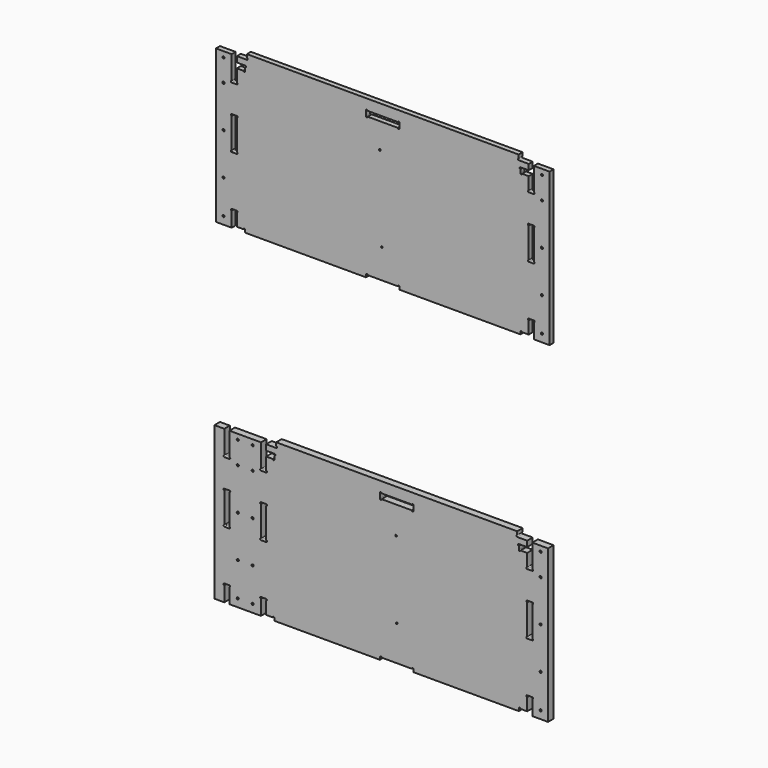
from build123d import *

# Parameters (mm, degrees)
F1_DEPTH = 18
F2_DEPTH = 25


# Not quite as in the source:
# - ends of sketch curves that miss each other by under 0.0002 mm in the source are joined


with BuildPart() as f1:
    # F0 (on Front) → F1 (new body)
    with BuildSketch(Plane.XZ):
        with BuildLine():
            Line((-599.985073, 1158.238852), (-599.999996, 608.956921))
            Line((-599.999996, 608.956921), (-543.499943, 608.956505))
            Line((-543.499943, 608.956505), (-543.499364, 662.686083))
            Line((-543.499364, 662.686083), (-543.499361, 662.91798))
            Line((-543.499361, 662.91798), (-543.730604, 662.935381))
            ThreePointArc((-543.730604, 662.935381), (-546.5166773993, 666.0571161852), (-543.4994899997, 668.9560841802))
            Line((-543.4994899997, 668.9560841802), (-524.999474, 668.955882))
            ThreePointArc((-524.999474, 668.955882), (-521.9913378584, 666.056393721), (-524.7686719668, 662.9351235758))
            Line((-524.7686719668, 662.9351235758), (-524.999155, 662.917071))
            Line((-524.999155, 662.917071), (-524.99915, 662.685882))
            Line((-524.99915, 662.685882), (-524.998175, 617.968196))
            Line((-524.998175, 617.968196), (-501.268235, 617.967938))
            Line((-501.268235, 617.967938), (-501.036338, 617.967935))
            Line((-501.036338, 617.967935), (-501.018937, 618.199178))
            ThreePointArc((-501.018937, 618.199178), (-497.8972013151, 620.9852513801), (-494.9982338214, 617.9680629997))
            Line((-494.9982338214, 617.9680629997), (-494.998333, 608.955947))
            Line((-494.998333, 608.955947), (-60.497611, 608.952295))
            Line((-60.497611, 608.952295), (-60.497513, 617.95625))
            ThreePointArc((-60.497513, 617.95625), (-57.5979261307, 620.9642909194), (-54.4767468993, 618.1868550079))
            Line((-54.4767468993, 618.1868550079), (-54.458702, 617.956372))
            Line((-54.458702, 617.956372), (-54.227513, 617.956369))
            Line((-54.227513, 617.956369), (53.732233, 617.955195))
            Line((53.732233, 617.955195), (53.964129, 617.955192))
            Line((53.964129, 617.955192), (53.981531, 618.186434))
            ThreePointArc((53.981531, 618.186434), (57.1032651816, 620.9725043987), (60.0022321834, 617.9553200013))
            Line((60.0022321834, 617.9553200013), (60.002404, 608.951))
            Line((60.002404, 608.951), (494.502793, 608.972372))
            Line((494.502793, 608.972372), (494.502859, 617.945383))
            ThreePointArc((494.502859, 617.945383), (497.4024353548, 620.9534335166), (500.5236242386, 618.1760090187))
            Line((500.5236242386, 618.1760090187), (500.54167, 617.945525))
            Line((500.54167, 617.945525), (500.772859, 617.945524))
            Line((500.772859, 617.945524), (524.502716, 617.945349))
            Line((524.502716, 617.945349), (524.501743, 662.671013))
            Line((524.501743, 662.671013), (524.501738, 662.902909))
            Line((524.501738, 662.902909), (524.270495, 662.920303))
            ThreePointArc((524.270495, 662.920303), (521.4843198384, 666.0419471329), (524.5014130005, 668.9410133346))
            Line((524.5014130005, 668.9410133346), (543.001446, 668.940811))
            ThreePointArc((543.001446, 668.940811), (546.0094849768, 666.0412236325), (543.232048014, 662.9200458215))
            Line((543.232048014, 662.9200458215), (543.001565, 662.902))
            Line((543.001565, 662.902), (543.001562, 662.670811))
            Line((543.001562, 662.670811), (543.000957, 608.948493))
            Line((543.000957, 608.948493), (599.50265, 608.948077))
            Line((599.50265, 608.948077), (599.515886, 1158.212743))
            Line((599.515886, 1158.212743), (543.016713, 1158.213833))
            Line((543.016713, 1158.213833), (543.013073, 1074.718273))
            Line((543.013073, 1074.718273), (543.013063, 1074.486377))
            Line((543.013063, 1074.486377), (543.244305, 1074.468968))
            ThreePointArc((543.244305, 1074.468968), (546.0302745941, 1071.3471417287), (543.012993, 1068.4482729774))
            Line((543.012993, 1068.4482729774), (524.514932, 1068.448531))
            ThreePointArc((524.514932, 1068.448531), (521.5069440099, 1071.3481709447), (524.2844350583, 1074.4693002551))
            Line((524.2844350583, 1074.4693002551), (524.514919, 1074.487342))
            Line((524.514919, 1074.487342), (524.514925, 1074.718531))
            Line((524.514925, 1074.718531), (524.516212, 1119.449306))
            Line((524.516212, 1119.449306), (500.786183, 1119.449822))
            Line((500.786183, 1119.449822), (500.554287, 1119.449827))
            Line((500.554287, 1119.449827), (500.536883, 1119.218585))
            ThreePointArc((500.536883, 1119.218585), (497.4151177731, 1116.4325458692), (494.5161828725, 1119.4497650002))
            Line((494.5161828725, 1119.4497650002), (494.51645, 1131.679977))
            Line((494.51645, 1131.679977), (494.516455, 1131.911873))
            Line((494.516455, 1131.911873), (494.285212, 1131.929277))
            ThreePointArc((494.285212, 1131.929277), (491.4991728692, 1135.0510422269), (494.5163920002, 1137.9499771275))
            Line((494.5163920002, 1137.9499771275), (524.516612, 1137.949324))
            Line((524.516612, 1137.949324), (524.516705, 1158.214243))
            Line((524.516705, 1158.214243), (488.515104, 1158.216167))
            ThreePointArc((488.515104, 1158.216167), (485.5070948152, 1161.1157859126), (488.2845650245, 1164.2369346868))
            Line((488.2845650245, 1164.2369346868), (488.515049, 1164.254978))
            Line((488.515049, 1164.254978), (488.515054, 1164.486167))
            Line((488.515054, 1164.486167), (488.515309, 1176.215177))
            Line((488.515309, 1176.215177), (-488.984612, 1176.236451))
            Line((-488.984612, 1176.236451), (-488.984867, 1164.507435))
            Line((-488.984867, 1164.507435), (-488.984872, 1164.275539))
            Line((-488.984872, 1164.275539), (-488.75363, 1164.258135))
            ThreePointArc((-488.75363, 1164.258135), (-485.9675908692, 1161.1363697731), (-488.9848100002, 1158.2374348725))
            Line((-488.9848100002, 1158.2374348725), (-524.984937, 1158.237949))
            Line((-524.984937, 1158.237949), (-524.985014, 1137.972314))
            Line((-524.985014, 1137.972314), (-494.985166, 1137.971661))
            ThreePointArc((-494.985166, 1137.971661), (-491.9771568152, 1135.0720420874), (-494.7546270245, 1131.9508933132))
            Line((-494.7546270245, 1131.9508933132), (-494.985111, 1131.93285))
            Line((-494.985111, 1131.93285), (-494.985116, 1131.701661))
            Line((-494.985116, 1131.701661), (-494.985382, 1119.47183))
            ThreePointArc((-494.985382, 1119.47183), (-497.8850009126, 1116.4638208152), (-501.0061496868, 1119.2412910245))
            Line((-501.0061496868, 1119.2412910245), (-501.024193, 1119.471774))
            Line((-501.024193, 1119.471774), (-501.255382, 1119.471779))
            Line((-501.255382, 1119.471779), (-524.985414, 1119.472296))
            Line((-524.985414, 1119.472296), (-524.986715, 1074.742245))
            Line((-524.986715, 1074.742245), (-524.986721, 1074.510349))
            Line((-524.986721, 1074.510349), (-524.755479, 1074.492943))
            ThreePointArc((-524.755479, 1074.492943), (-521.9694627151, 1071.3711577453), (-524.9867030001, 1068.4722449079))
            Line((-524.9867030001, 1068.4722449079), (-543.486726, 1068.472648))
            ThreePointArc((-543.486726, 1068.472648), (-546.4947351848, 1071.3722669126), (-543.7172649755, 1074.4934156868))
            Line((-543.7172649755, 1074.4934156868), (-543.486782, 1074.511459))
            Line((-543.486782, 1074.511459), (-543.486777, 1074.742648))
            Line((-543.486777, 1074.742648), (-543.48496, 1158.238346))
            Line((-543.48496, 1158.238346), (-599.985073, 1158.238852))
        make_face()
        with BuildLine():
            ThreePointArc((-572.840091, 640.229115), (-570.1884405706, 639.1307654294), (-569.090091, 636.479115))
            ThreePointArc((-569.090091, 636.479115), (-570.1884405706, 633.8274645706), (-572.840091, 632.729115))
            ThreePointArc((-572.840091, 632.729115), (-575.4917414294, 633.8274645706), (-576.590091, 636.479115))
            ThreePointArc((-576.590091, 636.479115), (-575.4917414294, 639.1307654294), (-572.840091, 640.229115))
        make_face(mode=Mode.SUBTRACT)
        with BuildLine():
            ThreePointArc((-572.840091, 761.929626), (-570.1884405706, 760.8312764294), (-569.090091, 758.179626))
            ThreePointArc((-569.090091, 758.179626), (-570.1884405706, 755.5279755706), (-572.840091, 754.429626))
            ThreePointArc((-572.840091, 754.429626), (-575.4917414294, 755.5279755706), (-576.590091, 758.179626))
            ThreePointArc((-576.590091, 758.179626), (-575.4917414294, 760.8312764294), (-572.840091, 761.929626))
        make_face(mode=Mode.SUBTRACT)
        with BuildLine():
            ThreePointArc((-572.840091, 911.929626), (-570.1884405706, 910.8312764294), (-569.090091, 908.179626))
            ThreePointArc((-569.090091, 908.179626), (-570.1884405706, 905.5279755706), (-572.840091, 904.429626))
            ThreePointArc((-572.840091, 904.429626), (-575.4917414294, 905.5279755706), (-576.590091, 908.179626))
            ThreePointArc((-576.590091, 908.179626), (-575.4917414294, 910.8312764294), (-572.840091, 911.929626))
        make_face(mode=Mode.SUBTRACT)
        with BuildLine():
            Line((-543.49218, 854.479583), (-543.491, 962.939703))
            ThreePointArc((-543.491, 962.9397030002), (-546.5009669998, 965.949736), (-543.490934, 968.9597029998))
            Line((-543.490934, 968.959703), (-524.990916, 968.959501))
            ThreePointArc((-524.990916, 968.9595009998), (-521.9809490002, 965.949468), (-524.990982, 962.9395010002))
            Line((-524.990982, 962.939501), (-524.992162, 854.479381))
            ThreePointArc((-524.992162, 854.4793809998), (-521.9821950002, 851.469348), (-524.992228, 848.4593810002))
            Line((-524.992228, 848.459381), (-543.492246, 848.459583))
            ThreePointArc((-543.492246, 848.4595830002), (-546.5022129998, 851.469616), (-543.49218, 854.4795829998))
        make_face(mode=Mode.SUBTRACT)
        with BuildLine():
            ThreePointArc((-572.840091, 1061.929626), (-570.1884405706, 1060.8312764294), (-569.090091, 1058.179626))
            ThreePointArc((-569.090091, 1058.179626), (-570.1884405706, 1055.5279755706), (-572.840091, 1054.429626))
            ThreePointArc((-572.840091, 1054.429626), (-575.4917414294, 1055.5279755706), (-576.590091, 1058.179626))
            ThreePointArc((-576.590091, 1058.179626), (-575.4917414294, 1060.8312764294), (-572.840091, 1061.929626))
        make_face(mode=Mode.SUBTRACT)
        with BuildLine():
            ThreePointArc((-572.840091, 1142.414271), (-570.1884405706, 1141.3159214294), (-569.090091, 1138.664271))
            ThreePointArc((-569.090091, 1138.664271), (-570.1884405706, 1136.0126205706), (-572.840091, 1134.914271))
            ThreePointArc((-572.840091, 1134.914271), (-575.4917414294, 1136.0126205706), (-576.590091, 1138.664271))
            ThreePointArc((-576.590091, 1138.664271), (-575.4917414294, 1141.3159214294), (-572.840091, 1142.414271))
        make_face(mode=Mode.SUBTRACT)
        with BuildLine():
            ThreePointArc((-6.303996, 722.984003), (-5.4253163436, 725.1053233436), (-3.303996, 725.984003))
            ThreePointArc((-3.303996, 725.984003), (-1.1826756564, 725.1053233436), (-0.303996, 722.984003))
            ThreePointArc((-0.303996, 722.984003), (-1.1826756564, 720.8626826564), (-3.303996, 719.984003))
            ThreePointArc((-3.303996, 719.984003), (-5.4253163436, 720.8626826564), (-6.303996, 722.984003))
        make_face(mode=Mode.SUBTRACT)
        Polygon((-36.965874, 892.758771), (-37.379663, 892.756003), (-37.799529, 892.752599), (-38.218499, 892.759839), (-38.636381, 892.777646), (-39.05298, 892.805945), (-39.468106, 892.84466), (-39.881563, 892.893716), (-40.29316, 892.953035), (-40.702704, 893.022544), (-41.110002, 893.102167), (-41.514861, 893.191826), (-41.917088, 893.291448), (-42.316491, 893.400956), (-42.712876, 893.520274), (-43.10605, 893.649328), (-43.495821, 893.78804), (-43.881996, 893.936336), (-44.264382, 894.09414), (-44.642786, 894.261376), (-45.017015, 894.437968), (-45.386876, 894.623841), (-45.752177, 894.818919), (-46.112725, 895.023127), (-46.468326, 895.236388), (-46.818788, 895.458628), (-47.163918, 895.689769), (-47.503523, 895.929738), (-47.83741, 896.178457), (-48.165387, 896.435852), (-48.48726, 896.701846), (-48.802837, 896.976364), (-49.111924, 897.25933), (-49.414329, 897.550669), (-49.76419, 897.930951), (-50.103711, 898.319139), (-50.432805, 898.715), (-50.751382, 899.1183), (-51.059353, 899.528805), (-51.35663, 899.946281), (-51.643124, 900.370494), (-51.918746, 900.801211), (-52.183407, 901.238197), (-52.437018, 901.681219), (-52.679491, 902.130043), (-52.910736, 902.584435), (-53.130664, 903.044161), (-53.339187, 903.508986), (-53.536217, 903.978678), (-53.721663, 904.453003), (-53.895437, 904.931725), (-54.057451, 905.414613), (-54.207614, 905.901431), (-54.34584, 906.391945), (-54.472038, 906.885923), (-54.58612, 907.38313), (-54.687997, 907.883331), (-54.777579, 908.386294), (-54.854779, 908.891785), (-54.919508, 909.399568), (-54.971676, 909.909412), (-55.011194, 910.421081), (-55.037974, 910.934342), (-55.051927, 911.44896), (-55.052964, 911.964703), (-55.040996, 912.481336), (-55.057067, 913.042457), (-55.058845, 913.602647), (-55.046428, 914.161646), (-55.019913, 914.719195), (-54.979398, 915.275036), (-54.92498, 915.828908), (-54.856758, 916.380553), (-54.774829, 916.929711), (-54.679291, 917.476123), (-54.570241, 918.019529), (-54.447777, 918.559671), (-54.311996, 919.096289), (-54.162997, 919.629124), (-54.000876, 920.157916), (-53.825732, 920.682407), (-53.637663, 921.202336), (-53.436765, 921.717445), (-53.223137, 922.227475), (-52.996876, 922.732165), (-52.758079, 923.231258), (-52.506846, 923.724493), (-52.243272, 924.211611), (-51.967456, 924.692354), (-51.679496, 925.166461), (-51.379489, 925.633674), (-51.067533, 926.093733), (-50.743725, 926.546378), (-50.408163, 926.991352), (-50.060945, 927.428393), (-49.702168, 927.857244), (-49.33193, 928.277645), (-48.950329, 928.689336), (-48.664581, 928.98001), (-48.371965, 929.262477), (-48.072679, 929.536657), (-47.766918, 929.802466), (-47.454877, 930.059825), (-47.136753, 930.30865), (-46.812741, 930.548862), (-46.483038, 930.780378), (-46.147838, 931.003116), (-45.807338, 931.216996), (-45.461733, 931.421935), (-45.11122, 931.617852), (-44.755994, 931.804665), (-44.396251, 931.982294), (-44.032186, 932.150656), (-43.663996, 932.309669), (-43.291876, 932.459253), (-42.916023, 932.599326), (-42.536631, 932.729806), (-42.153897, 932.850612), (-41.768017, 932.961662), (-41.379186, 933.062874), (-40.9876, 933.154168), (-40.593454, 933.235461), (-40.196946, 933.306672), (-39.79827, 933.367719), (-39.397623, 933.418522), (-38.995199, 933.458997), (-38.591196, 933.489065), (-38.185808, 933.508643), (-37.779232, 933.517649), (-37.371663, 933.516003), (-36.957415, 933.512329), (-36.544302, 933.497865), (-36.132524, 933.472695), (-35.722277, 933.436904), (-35.313762, 933.390575), (-34.907174, 933.333794), (-34.502714, 933.266644), (-34.100579, 933.189211), (-33.700968, 933.101579), (-33.304078, 933.003831), (-32.910108, 932.896054), (-32.519257, 932.778331), (-32.131721, 932.650746), (-31.747701, 932.513385), (-31.367393, 932.366331), (-30.990996, 932.209669), (-30.618709, 932.043484), (-30.250729, 931.86786), (-29.887255, 931.682882), (-29.528486, 931.488633), (-29.174618, 931.285199), (-28.825852, 931.072663), (-28.482384, 930.851112), (-28.144413, 930.620628), (-27.812137, 930.381296), (-27.485755, 930.133201), (-27.165465, 929.876428), (-26.851465, 929.61106), (-26.543953, 929.337182), (-26.243128, 929.05488), (-25.949187, 928.764236), (-25.662329, 928.465336), (-25.292149, 928.055808), (-24.933171, 927.637893), (-24.585485, 927.211844), (-24.249184, 926.777914), (-23.924359, 926.336358), (-23.611103, 925.887428), (-23.309507, 925.431378), (-23.019663, 924.968461), (-22.741662, 924.498931), (-22.475598, 924.023041), (-22.22156, 923.541045), (-21.979642, 923.053195), (-21.749935, 922.559746), (-21.53253, 922.060951), (-21.32752, 921.557063), (-21.134996, 921.048336), (-20.95505, 920.535023), (-20.787775, 920.017377), (-20.633261, 919.495652), (-20.4916, 918.970102), (-20.362885, 918.440979), (-20.247207, 917.908537), (-20.144658, 917.37303), (-20.055329, 916.834711), (-19.979313, 916.293833), (-19.916702, 915.75065), (-19.867586, 915.205416), (-19.832059, 914.658383), (-19.810211, 914.109805), (-19.802134, 913.559936), (-19.807921, 913.009028), (-19.827663, 912.457336), (-19.819233, 911.942508), (-19.823884, 911.428683), (-19.841523, 910.916097), (-19.872059, 910.404987), (-19.915399, 909.89559), (-19.971452, 909.388143), (-20.040126, 908.882882), (-20.121329, 908.380044), (-20.21497, 907.879867), (-20.320957, 907.382587), (-20.439198, 906.88844), (-20.5696, 906.397664), (-20.712073, 905.910496), (-20.866525, 905.427171), (-21.032863, 904.947928), (-21.210996, 904.473003), (-21.400832, 904.002632), (-21.60228, 903.537053), (-21.815247, 903.076502), (-22.039642, 902.621216), (-22.275373, 902.171432), (-22.522348, 901.727387), (-22.780475, 901.289318), (-23.049663, 900.857461), (-23.329819, 900.432053), (-23.620853, 900.013331), (-23.922672, 899.601533), (-24.235184, 899.196893), (-24.558297, 898.799651), (-24.891921, 898.410041), (-25.235962, 898.028302), (-25.590329, 897.654669), (-25.884236, 897.363456), (-26.184829, 897.080368), (-26.491921, 896.805484), (-26.805324, 896.538883), (-27.12485, 896.280643), (-27.450312, 896.030843), (-27.78152, 895.789562), (-28.118288, 895.556878), (-28.460426, 895.332869), (-28.807748, 895.117615), (-29.160065, 894.911194), (-29.517189, 894.713685), (-29.878932, 894.525166), (-30.245106, 894.345716), (-30.615524, 894.175413), (-30.989996, 894.014336), (-31.368336, 893.862564), (-31.750355, 893.720175), (-32.135865, 893.587248), (-32.524678, 893.463862), (-32.916607, 893.350095), (-33.311463, 893.246025), (-33.709058, 893.151732), (-34.109204, 893.067294), (-34.511714, 892.99279), (-34.916399, 892.928298), (-35.323071, 892.873896), (-35.731543, 892.829664), (-36.141626, 892.79568), (-36.553132, 892.772023), align=None, mode=Mode.SUBTRACT)
        with BuildLine():
            ThreePointArc((-13.994996, 1028.710003), (-13.1163163436, 1030.8313233436), (-10.994996, 1031.710003))
            ThreePointArc((-10.994996, 1031.710003), (-8.8736756564, 1030.8313233436), (-7.994996, 1028.710003))
            ThreePointArc((-7.994996, 1028.710003), (-8.8736756564, 1026.5886826564), (-10.994996, 1025.710003))
            ThreePointArc((-10.994996, 1025.710003), (-13.1163163436, 1026.5886826564), (-13.994996, 1028.710003))
        make_face(mode=Mode.SUBTRACT)
        Polygon((7.27946, 892.758771), (6.865671, 892.756003), (6.445804, 892.752599), (6.026834, 892.759839), (5.608953, 892.777646), (5.192353, 892.805945), (4.777228, 892.84466), (4.36377, 892.893716), (3.952173, 892.953035), (3.542629, 893.022544), (3.135331, 893.102167), (2.730472, 893.191826), (2.328245, 893.291448), (1.928842, 893.400956), (1.532458, 893.520274), (1.139283, 893.649328), (0.749512, 893.78804), (0.363337, 893.936336), (-0.019049, 894.09414), (-0.397452, 894.261376), (-0.771682, 894.437968), (-1.141543, 894.623841), (-1.506844, 894.818919), (-1.867391, 895.023127), (-2.222992, 895.236388), (-2.573454, 895.458628), (-2.918584, 895.689769), (-3.258189, 895.929738), (-3.592077, 896.178457), (-3.920053, 896.435852), (-4.241927, 896.701846), (-4.557503, 896.976364), (-4.866591, 897.25933), (-5.168996, 897.550669), (-5.518856, 897.930951), (-5.858378, 898.319139), (-6.187471, 898.715), (-6.506048, 899.1183), (-6.81402, 899.528805), (-7.111297, 899.946281), (-7.397791, 900.370494), (-7.673413, 900.801211), (-7.938074, 901.238197), (-8.191685, 901.681219), (-8.434157, 902.130043), (-8.665402, 902.584435), (-8.885331, 903.044161), (-9.093854, 903.508986), (-9.290883, 903.978678), (-9.476329, 904.453003), (-9.650104, 904.931725), (-9.812117, 905.414613), (-9.962281, 905.901431), (-10.100507, 906.391945), (-10.226705, 906.885923), (-10.340786, 907.38313), (-10.442663, 907.883331), (-10.532246, 908.386294), (-10.609446, 908.891785), (-10.674174, 909.399568), (-10.726342, 909.909412), (-10.765861, 910.421081), (-10.792641, 910.934342), (-10.806594, 911.44896), (-10.807631, 911.964703), (-10.795663, 912.481336), (-10.811734, 913.042457), (-10.813512, 913.602647), (-10.801094, 914.161646), (-10.774579, 914.719195), (-10.734064, 915.275036), (-10.679647, 915.828908), (-10.611425, 916.380553), (-10.529496, 916.929711), (-10.433958, 917.476123), (-10.324908, 918.019529), (-10.202443, 918.559671), (-10.066663, 919.096289), (-9.917663, 919.629124), (-9.755543, 920.157916), (-9.580399, 920.682407), (-9.392329, 921.202336), (-9.191432, 921.717445), (-8.977803, 922.227475), (-8.751542, 922.732165), (-8.512746, 923.231258), (-8.261512, 923.724493), (-7.997939, 924.211611), (-7.722123, 924.692354), (-7.434163, 925.166461), (-7.134156, 925.633674), (-6.822199, 926.093733), (-6.498391, 926.546378), (-6.162829, 926.991352), (-5.815611, 927.428393), (-5.456835, 927.857244), (-5.086597, 928.277645), (-4.704996, 928.689336), (-4.419247, 928.98001), (-4.126632, 929.262477), (-3.827346, 929.536657), (-3.521585, 929.802466), (-3.209544, 930.059825), (-2.89142, 930.30865), (-2.567408, 930.548862), (-2.237704, 930.780378), (-1.902505, 931.003116), (-1.562005, 931.216996), (-1.2164, 931.421935), (-0.865887, 931.617852), (-0.510661, 931.804665), (-0.150917, 931.982294), (0.213147, 932.150656), (0.581337, 932.309669), (0.953457, 932.459253), (1.329311, 932.599326), (1.708702, 932.729806), (2.091436, 932.850612), (2.477317, 932.961662), (2.866148, 933.062874), (3.257734, 933.154168), (3.651879, 933.235461), (4.048387, 933.306672), (4.447063, 933.367719), (4.847711, 933.418522), (5.250134, 933.458997), (5.654138, 933.489065), (6.059525, 933.508643), (6.466102, 933.517649), (6.873671, 933.516003), (7.287919, 933.512329), (7.701031, 933.497865), (8.11281, 933.472695), (8.523056, 933.436904), (8.931572, 933.390575), (9.338159, 933.333794), (9.742619, 933.266644), (10.144754, 933.189211), (10.544365, 933.101579), (10.941255, 933.003831), (11.335225, 932.896054), (11.726077, 932.778331), (12.113612, 932.650746), (12.497633, 932.513385), (12.877941, 932.366331), (13.254337, 932.209669), (13.626625, 932.043484), (13.994604, 931.86786), (14.358078, 931.682882), (14.716848, 931.488633), (15.070715, 931.285199), (15.419482, 931.072663), (15.76295, 930.851112), (16.100921, 930.620628), (16.433196, 930.381296), (16.759578, 930.133201), (17.079868, 929.876428), (17.393868, 929.61106), (17.70138, 929.337182), (18.002206, 929.05488), (18.296146, 928.764236), (18.583004, 928.465336), (18.953184, 928.055808), (19.312163, 927.637893), (19.659849, 927.211844), (19.99615, 926.777914), (20.320974, 926.336358), (20.63423, 925.887428), (20.935827, 925.431378), (21.225671, 924.968461), (21.503671, 924.498931), (21.769736, 924.023041), (22.023773, 923.541045), (22.265691, 923.053195), (22.495399, 922.559746), (22.712803, 922.060951), (22.917813, 921.557063), (23.110337, 921.048336), (23.290283, 920.535023), (23.457559, 920.017377), (23.612073, 919.495652), (23.753733, 918.970102), (23.882448, 918.440979), (23.998126, 917.908537), (24.100675, 917.37303), (24.190004, 916.834711), (24.26602, 916.293833), (24.328632, 915.75065), (24.377747, 915.205416), (24.413275, 914.658383), (24.435123, 914.109805), (24.443199, 913.559936), (24.437412, 913.009028), (24.417671, 912.457336), (24.4261, 911.942508), (24.421449, 911.428683), (24.40381, 910.916097), (24.373275, 910.404987), (24.329935, 909.89559), (24.273882, 909.388143), (24.205207, 908.882882), (24.124004, 908.380044), (24.030363, 907.879867), (23.924376, 907.382587), (23.806136, 906.88844), (23.675733, 906.397664), (23.53326, 905.910496), (23.378809, 905.427171), (23.21247, 904.947928), (23.034337, 904.473003), (22.844501, 904.002632), (22.643053, 903.537053), (22.430086, 903.076502), (22.205691, 902.621216), (21.969961, 902.171432), (21.722986, 901.727387), (21.464858, 901.289318), (21.195671, 900.857461), (20.915514, 900.432053), (20.62448, 900.013331), (20.322662, 899.601533), (20.01015, 899.196893), (19.687036, 898.799651), (19.353413, 898.410041), (19.009371, 898.028302), (18.655004, 897.654669), (18.361098, 897.363456), (18.060505, 897.080368), (17.753412, 896.805484), (17.440009, 896.538883), (17.120483, 896.280643), (16.795021, 896.030843), (16.463813, 895.789562), (16.127046, 895.556878), (15.784907, 895.332869), (15.437585, 895.117615), (15.085268, 894.911194), (14.728145, 894.713685), (14.366401, 894.525166), (14.000227, 894.345716), (13.62981, 894.175413), (13.255337, 894.014336), (12.876997, 893.862564), (12.494979, 893.720175), (12.109468, 893.587248), (11.720655, 893.463862), (11.328726, 893.350095), (10.93387, 893.246025), (10.536275, 893.151732), (10.136129, 893.067294), (9.733619, 892.99279), (9.328934, 892.928298), (8.922262, 892.873896), (8.51379, 892.829664), (8.103707, 892.79568), (7.692201, 892.772023), align=None, mode=Mode.SUBTRACT)
        Polygon((50.999004, 913.305336), (33.441671, 913.305336), (33.441671, 933.276003), (50.999004, 933.276003), (51.49338, 933.272599), (51.984884, 933.243649), (52.472584, 933.189542), (52.955546, 933.110669), (53.432835, 933.007422), (53.90352, 932.88019), (54.366665, 932.729365), (54.821337, 932.555336), (55.266604, 932.358495), (55.70153, 932.139232), (56.125183, 931.897938), (56.536629, 931.635003), (56.934934, 931.350818), (57.319165, 931.045774), (57.688389, 930.720261), (58.041671, 930.374669), (58.382109, 930.023162), (58.703181, 929.656232), (59.004518, 929.274771), (59.285754, 928.879669), (59.546521, 928.471818), (59.786452, 928.052107), (60.00518, 927.621427), (60.202337, 927.180669), (60.377557, 926.730724), (60.530473, 926.272482), (60.660716, 925.806833), (60.767921, 925.334669), (60.851719, 924.85688), (60.911743, 924.374357), (60.947628, 923.88799), (60.959004, 923.398669), (60.961973, 922.897108), (60.939134, 922.398055), (60.890865, 921.902455), (60.817546, 921.411253), (60.719554, 920.925395), (60.59727, 920.445826), (60.451071, 919.973491), (60.281337, 919.509336), (60.088447, 919.054306), (59.87278, 918.609346), (59.634714, 918.175402), (59.374629, 917.753419), (59.092903, 917.344343), (58.789915, 916.949117), (58.466045, 916.568689), (58.121671, 916.204003), (57.761543, 915.859877), (57.385775, 915.535747), (56.995288, 915.231985), (56.591004, 914.948961), (56.173845, 914.687046), (55.744733, 914.446612), (55.30459, 914.228029), (54.854337, 914.031669), (54.394897, 913.857903), (53.927191, 913.707102), (53.452142, 913.579636), (52.970671, 913.475878), (52.483699, 913.396197), (51.99215, 913.340966), (51.496944, 913.310555), align=None, mode=Mode.SUBTRACT)
        with BuildLine():
            Line((53.99369, 1119.459988), (-54.46643, 1119.462349))
            ThreePointArc((-54.4664300007, 1119.462349), (-57.4764955, 1116.4524140007), (-60.4864299993, 1119.46248))
            Line((-60.48643, 1119.46248), (-60.486028, 1137.962498))
            ThreePointArc((-60.4860279993, 1137.962498), (-57.4759625, 1140.9724329993), (-54.4660280007, 1137.962367))
            Line((-54.466028, 1137.962367), (53.994092, 1137.960006))
            ThreePointArc((53.9940920007, 1137.960006), (57.0041575, 1140.9699399993), (60.0140919993, 1137.959875))
            Line((60.014092, 1137.959875), (60.01369, 1119.459857))
            ThreePointArc((60.0136899993, 1119.459857), (57.0036245, 1116.4499230007), (53.9936900007, 1119.459988))
        make_face(mode=Mode.SUBTRACT)
        with BuildLine():
            ThreePointArc((571.966185, 640.229115), (574.6178354294, 639.1307654294), (575.716185, 636.479115))
            ThreePointArc((575.716185, 636.479115), (574.6178354294, 633.8274645706), (571.966185, 632.729115))
            ThreePointArc((571.966185, 632.729115), (569.3145345706, 633.8274645706), (568.216185, 636.479115))
            ThreePointArc((568.216185, 636.479115), (569.3145345706, 639.1307654294), (571.966185, 640.229115))
        make_face(mode=Mode.SUBTRACT)
        with BuildLine():
            ThreePointArc((571.966185, 761.929626), (574.6178354294, 760.8312764294), (575.716185, 758.179626))
            ThreePointArc((575.716185, 758.179626), (574.6178354294, 755.5279755706), (571.966185, 754.429626))
            ThreePointArc((571.966185, 754.429626), (569.3145345706, 755.5279755706), (568.216185, 758.179626))
            ThreePointArc((568.216185, 758.179626), (569.3145345706, 760.8312764294), (571.966185, 761.929626))
        make_face(mode=Mode.SUBTRACT)
        with BuildLine():
            Line((543.008673, 848.448946), (524.50888, 848.449147))
            ThreePointArc((524.50888, 848.4491470002), (521.4989130002, 851.45918), (524.508946, 854.4691469998))
            Line((524.508946, 854.469147), (524.510126, 962.929319))
            ThreePointArc((524.510126, 962.9293190002), (521.5001580002, 965.9393515), (524.510191, 968.9493189998))
            Line((524.510191, 968.949319), (543.009985, 968.949113))
            ThreePointArc((543.009985, 968.9491129998), (546.0199519998, 965.93908), (543.009919, 962.9291130002))
            Line((543.009919, 962.929113), (543.008739, 854.468946))
            ThreePointArc((543.008739, 854.4689459998), (546.0187059998, 851.458913), (543.008673, 848.4489460002))
        make_face(mode=Mode.SUBTRACT)
        with BuildLine():
            ThreePointArc((571.966185, 911.929626), (574.6178354294, 910.8312764294), (575.716185, 908.179626))
            ThreePointArc((575.716185, 908.179626), (574.6178354294, 905.5279755706), (571.966185, 904.429626))
            ThreePointArc((571.966185, 904.429626), (569.3145345706, 905.5279755706), (568.216185, 908.179626))
            ThreePointArc((568.216185, 908.179626), (569.3145345706, 910.8312764294), (571.966185, 911.929626))
        make_face(mode=Mode.SUBTRACT)
        with BuildLine():
            ThreePointArc((571.966185, 1061.929626), (574.6178354294, 1060.8312764294), (575.716185, 1058.179626))
            ThreePointArc((575.716185, 1058.179626), (574.6178354294, 1055.5279755706), (571.966185, 1054.429626))
            ThreePointArc((571.966185, 1054.429626), (569.3145345706, 1055.5279755706), (568.216185, 1058.179626))
            ThreePointArc((568.216185, 1058.179626), (569.3145345706, 1060.8312764294), (571.966185, 1061.929626))
        make_face(mode=Mode.SUBTRACT)
        with BuildLine():
            ThreePointArc((571.966185, 1142.414271), (574.6178354294, 1141.3159214294), (575.716185, 1138.664271))
            ThreePointArc((575.716185, 1138.664271), (574.6178354294, 1136.0126205706), (571.966185, 1134.914271))
            ThreePointArc((571.966185, 1134.914271), (569.3145345706, 1136.0126205706), (568.216185, 1138.664271))
            ThreePointArc((568.216185, 1138.664271), (569.3145345706, 1141.3159214294), (571.966185, 1142.414271))
        make_face(mode=Mode.SUBTRACT)
        Polygon((-37.799529, 892.752599), (-37.379663, 892.756003), (-36.965874, 892.758771), (-36.553132, 892.772023), (-36.141626, 892.79568), (-35.731543, 892.829664), (-35.323071, 892.873896), (-34.916399, 892.928298), (-34.511714, 892.99279), (-34.109204, 893.067294), (-33.709058, 893.151732), (-33.311463, 893.246025), (-32.916607, 893.350095), (-32.524678, 893.463862), (-32.135865, 893.587248), (-31.750355, 893.720175), (-31.368336, 893.862564), (-30.989996, 894.014336), (-30.615524, 894.175413), (-30.245106, 894.345716), (-29.878932, 894.525166), (-29.517189, 894.713685), (-29.160065, 894.911194), (-28.807748, 895.117615), (-28.460426, 895.332869), (-28.118288, 895.556878), (-27.78152, 895.789562), (-27.450312, 896.030843), (-27.12485, 896.280643), (-26.805324, 896.538883), (-26.491921, 896.805484), (-26.184829, 897.080368), (-25.884236, 897.363456), (-25.590329, 897.654669), (-25.235962, 898.028302), (-24.891921, 898.410041), (-24.558297, 898.799651), (-24.235184, 899.196893), (-23.922672, 899.601533), (-23.620853, 900.013331), (-23.329819, 900.432053), (-23.049663, 900.857461), (-22.780475, 901.289318), (-22.522348, 901.727387), (-22.275373, 902.171432), (-22.039642, 902.621216), (-21.815247, 903.076502), (-21.60228, 903.537053), (-21.400832, 904.002632), (-21.210996, 904.473003), (-21.032863, 904.947928), (-20.866525, 905.427171), (-20.712073, 905.910496), (-20.5696, 906.397664), (-20.439198, 906.88844), (-20.320957, 907.382587), (-20.21497, 907.879867), (-20.121329, 908.380044), (-20.040126, 908.882882), (-19.971452, 909.388143), (-19.915399, 909.89559), (-19.872059, 910.404987), (-19.841523, 910.916097), (-19.823884, 911.428683), (-19.819233, 911.942508), (-19.827663, 912.457336), (-19.807921, 913.009028), (-19.802134, 913.559936), (-19.810211, 914.109805), (-19.832059, 914.658383), (-19.867586, 915.205416), (-19.916702, 915.75065), (-19.979313, 916.293833), (-20.055329, 916.834711), (-20.144658, 917.37303), (-20.247207, 917.908537), (-20.362885, 918.440979), (-20.4916, 918.970102), (-20.633261, 919.495652), (-20.787775, 920.017377), (-20.95505, 920.535023), (-21.134996, 921.048336), (-21.32752, 921.557063), (-21.53253, 922.060951), (-21.749935, 922.559746), (-21.979642, 923.053195), (-22.22156, 923.541045), (-22.475598, 924.023041), (-22.741662, 924.498931), (-23.019663, 924.968461), (-23.309507, 925.431378), (-23.611103, 925.887428), (-23.924359, 926.336358), (-24.249184, 926.777914), (-24.585485, 927.211844), (-24.933171, 927.637893), (-25.292149, 928.055808), (-25.662329, 928.465336), (-25.949187, 928.764236), (-26.243128, 929.05488), (-26.543953, 929.337182), (-26.851465, 929.61106), (-27.165465, 929.876428), (-27.485755, 930.133201), (-27.812137, 930.381296), (-28.144413, 930.620628), (-28.482384, 930.851112), (-28.825852, 931.072663), (-29.174618, 931.285199), (-29.528486, 931.488633), (-29.887255, 931.682882), (-30.250729, 931.86786), (-30.618709, 932.043484), (-30.990996, 932.209669), (-31.367393, 932.366331), (-31.747701, 932.513385), (-32.131721, 932.650746), (-32.519257, 932.778331), (-32.910108, 932.896054), (-33.304078, 933.003831), (-33.700968, 933.101579), (-34.100579, 933.189211), (-34.502714, 933.266644), (-34.907174, 933.333794), (-35.313762, 933.390575), (-35.722277, 933.436904), (-36.132524, 933.472695), (-36.544302, 933.497865), (-36.957415, 933.512329), (-37.371663, 933.516003), (-37.779232, 933.517649), (-38.185808, 933.508643), (-38.591196, 933.489065), (-38.995199, 933.458997), (-39.397623, 933.418522), (-39.79827, 933.367719), (-40.196946, 933.306672), (-40.593454, 933.235461), (-40.9876, 933.154168), (-41.379186, 933.062874), (-41.768017, 932.961662), (-42.153897, 932.850612), (-42.536631, 932.729806), (-42.916023, 932.599326), (-43.291876, 932.459253), (-43.663996, 932.309669), (-44.032186, 932.150656), (-44.396251, 931.982294), (-44.755994, 931.804665), (-45.11122, 931.617852), (-45.461733, 931.421935), (-45.807338, 931.216996), (-46.147838, 931.003116), (-46.483038, 930.780378), (-46.812741, 930.548862), (-47.136753, 930.30865), (-47.454877, 930.059825), (-47.766918, 929.802466), (-48.072679, 929.536657), (-48.371965, 929.262477), (-48.664581, 928.98001), (-48.950329, 928.689336), (-49.33193, 928.277645), (-49.702168, 927.857244), (-50.060945, 927.428393), (-50.408163, 926.991352), (-50.743725, 926.546378), (-51.067533, 926.093733), (-51.379489, 925.633674), (-51.679496, 925.166461), (-51.967456, 924.692354), (-52.243272, 924.211611), (-52.506846, 923.724493), (-52.758079, 923.231258), (-52.996876, 922.732165), (-53.223137, 922.227475), (-53.436765, 921.717445), (-53.637663, 921.202336), (-53.825732, 920.682407), (-54.000876, 920.157916), (-54.162997, 919.629124), (-54.311996, 919.096289), (-54.447777, 918.559671), (-54.570241, 918.019529), (-54.679291, 917.476123), (-54.774829, 916.929711), (-54.856758, 916.380553), (-54.92498, 915.828908), (-54.979398, 915.275036), (-55.019913, 914.719195), (-55.046428, 914.161646), (-55.058845, 913.602647), (-55.057067, 913.042457), (-55.040996, 912.481336), (-55.052964, 911.964703), (-55.051927, 911.44896), (-55.037974, 910.934342), (-55.011194, 910.421081), (-54.971676, 909.909412), (-54.919508, 909.399568), (-54.854779, 908.891785), (-54.777579, 908.386294), (-54.687997, 907.883331), (-54.58612, 907.38313), (-54.472038, 906.885923), (-54.34584, 906.391945), (-54.207614, 905.901431), (-54.057451, 905.414613), (-53.895437, 904.931725), (-53.721663, 904.453003), (-53.536217, 903.978678), (-53.339187, 903.508986), (-53.130664, 903.044161), (-52.910736, 902.584435), (-52.679491, 902.130043), (-52.437018, 901.681219), (-52.183407, 901.238197), (-51.918746, 900.801211), (-51.643124, 900.370494), (-51.35663, 899.946281), (-51.059353, 899.528805), (-50.751382, 899.1183), (-50.432805, 898.715), (-50.103711, 898.319139), (-49.76419, 897.930951), (-49.414329, 897.550669), (-49.111924, 897.25933), (-48.802837, 896.976364), (-48.48726, 896.701846), (-48.165387, 896.435852), (-47.83741, 896.178457), (-47.503523, 895.929738), (-47.163918, 895.689769), (-46.818788, 895.458628), (-46.468326, 895.236388), (-46.112725, 895.023127), (-45.752177, 894.818919), (-45.386876, 894.623841), (-45.017015, 894.437968), (-44.642786, 894.261376), (-44.264382, 894.09414), (-43.881996, 893.936336), (-43.495821, 893.78804), (-43.10605, 893.649328), (-42.712876, 893.520274), (-42.316491, 893.400956), (-41.917088, 893.291448), (-41.514861, 893.191826), (-41.110002, 893.102167), (-40.702704, 893.022544), (-40.29316, 892.953035), (-39.881563, 892.893716), (-39.468106, 892.84466), (-39.05298, 892.805945), (-38.636381, 892.777646), (-38.218499, 892.759839), align=None)
        Polygon((6.445804, 892.752599), (6.865671, 892.756003), (7.27946, 892.758771), (7.692201, 892.772023), (8.103707, 892.79568), (8.51379, 892.829664), (8.922262, 892.873896), (9.328934, 892.928298), (9.733619, 892.99279), (10.136129, 893.067294), (10.536275, 893.151732), (10.93387, 893.246025), (11.328726, 893.350095), (11.720655, 893.463862), (12.109468, 893.587248), (12.494979, 893.720175), (12.876997, 893.862564), (13.255337, 894.014336), (13.62981, 894.175413), (14.000227, 894.345716), (14.366401, 894.525166), (14.728145, 894.713685), (15.085268, 894.911194), (15.437585, 895.117615), (15.784907, 895.332869), (16.127046, 895.556878), (16.463813, 895.789562), (16.795021, 896.030843), (17.120483, 896.280643), (17.440009, 896.538883), (17.753412, 896.805484), (18.060505, 897.080368), (18.361098, 897.363456), (18.655004, 897.654669), (19.009371, 898.028302), (19.353413, 898.410041), (19.687036, 898.799651), (20.01015, 899.196893), (20.322662, 899.601533), (20.62448, 900.013331), (20.915514, 900.432053), (21.195671, 900.857461), (21.464858, 901.289318), (21.722986, 901.727387), (21.969961, 902.171432), (22.205691, 902.621216), (22.430086, 903.076502), (22.643053, 903.537053), (22.844501, 904.002632), (23.034337, 904.473003), (23.21247, 904.947928), (23.378809, 905.427171), (23.53326, 905.910496), (23.675733, 906.397664), (23.806136, 906.88844), (23.924376, 907.382587), (24.030363, 907.879867), (24.124004, 908.380044), (24.205207, 908.882882), (24.273882, 909.388143), (24.329935, 909.89559), (24.373275, 910.404987), (24.40381, 910.916097), (24.421449, 911.428683), (24.4261, 911.942508), (24.417671, 912.457336), (24.437412, 913.009028), (24.443199, 913.559936), (24.435123, 914.109805), (24.413275, 914.658383), (24.377747, 915.205416), (24.328632, 915.75065), (24.26602, 916.293833), (24.190004, 916.834711), (24.100675, 917.37303), (23.998126, 917.908537), (23.882448, 918.440979), (23.753733, 918.970102), (23.612073, 919.495652), (23.457559, 920.017377), (23.290283, 920.535023), (23.110337, 921.048336), (22.917813, 921.557063), (22.712803, 922.060951), (22.495399, 922.559746), (22.265691, 923.053195), (22.023773, 923.541045), (21.769736, 924.023041), (21.503671, 924.498931), (21.225671, 924.968461), (20.935827, 925.431378), (20.63423, 925.887428), (20.320974, 926.336358), (19.99615, 926.777914), (19.659849, 927.211844), (19.312163, 927.637893), (18.953184, 928.055808), (18.583004, 928.465336), (18.296146, 928.764236), (18.002206, 929.05488), (17.70138, 929.337182), (17.393868, 929.61106), (17.079868, 929.876428), (16.759578, 930.133201), (16.433196, 930.381296), (16.100921, 930.620628), (15.76295, 930.851112), (15.419482, 931.072663), (15.070715, 931.285199), (14.716848, 931.488633), (14.358078, 931.682882), (13.994604, 931.86786), (13.626625, 932.043484), (13.254337, 932.209669), (12.877941, 932.366331), (12.497633, 932.513385), (12.113612, 932.650746), (11.726077, 932.778331), (11.335225, 932.896054), (10.941255, 933.003831), (10.544365, 933.101579), (10.144754, 933.189211), (9.742619, 933.266644), (9.338159, 933.333794), (8.931572, 933.390575), (8.523056, 933.436904), (8.11281, 933.472695), (7.701031, 933.497865), (7.287919, 933.512329), (6.873671, 933.516003), (6.466102, 933.517649), (6.059525, 933.508643), (5.654138, 933.489065), (5.250134, 933.458997), (4.847711, 933.418522), (4.447063, 933.367719), (4.048387, 933.306672), (3.651879, 933.235461), (3.257734, 933.154168), (2.866148, 933.062874), (2.477317, 932.961662), (2.091436, 932.850612), (1.708702, 932.729806), (1.329311, 932.599326), (0.953457, 932.459253), (0.581337, 932.309669), (0.213147, 932.150656), (-0.150917, 931.982294), (-0.510661, 931.804665), (-0.865887, 931.617852), (-1.2164, 931.421935), (-1.562005, 931.216996), (-1.902505, 931.003116), (-2.237704, 930.780378), (-2.567408, 930.548862), (-2.89142, 930.30865), (-3.209544, 930.059825), (-3.521585, 929.802466), (-3.827346, 929.536657), (-4.126632, 929.262477), (-4.419247, 928.98001), (-4.704996, 928.689336), (-5.086597, 928.277645), (-5.456835, 927.857244), (-5.815611, 927.428393), (-6.162829, 926.991352), (-6.498391, 926.546378), (-6.822199, 926.093733), (-7.134156, 925.633674), (-7.434163, 925.166461), (-7.722123, 924.692354), (-7.997939, 924.211611), (-8.261512, 923.724493), (-8.512746, 923.231258), (-8.751542, 922.732165), (-8.977803, 922.227475), (-9.191432, 921.717445), (-9.392329, 921.202336), (-9.580399, 920.682407), (-9.755543, 920.157916), (-9.917663, 919.629124), (-10.066663, 919.096289), (-10.202443, 918.559671), (-10.324908, 918.019529), (-10.433958, 917.476123), (-10.529496, 916.929711), (-10.611425, 916.380553), (-10.679647, 915.828908), (-10.734064, 915.275036), (-10.774579, 914.719195), (-10.801094, 914.161646), (-10.813512, 913.602647), (-10.811734, 913.042457), (-10.795663, 912.481336), (-10.807631, 911.964703), (-10.806594, 911.44896), (-10.792641, 910.934342), (-10.765861, 910.421081), (-10.726342, 909.909412), (-10.674174, 909.399568), (-10.609446, 908.891785), (-10.532246, 908.386294), (-10.442663, 907.883331), (-10.340786, 907.38313), (-10.226705, 906.885923), (-10.100507, 906.391945), (-9.962281, 905.901431), (-9.812117, 905.414613), (-9.650104, 904.931725), (-9.476329, 904.453003), (-9.290883, 903.978678), (-9.093854, 903.508986), (-8.885331, 903.044161), (-8.665402, 902.584435), (-8.434157, 902.130043), (-8.191685, 901.681219), (-7.938074, 901.238197), (-7.673413, 900.801211), (-7.397791, 900.370494), (-7.111297, 899.946281), (-6.81402, 899.528805), (-6.506048, 899.1183), (-6.187471, 898.715), (-5.858378, 898.319139), (-5.518856, 897.930951), (-5.168996, 897.550669), (-4.866591, 897.25933), (-4.557503, 896.976364), (-4.241927, 896.701846), (-3.920053, 896.435852), (-3.592077, 896.178457), (-3.258189, 895.929738), (-2.918584, 895.689769), (-2.573454, 895.458628), (-2.222992, 895.236388), (-1.867391, 895.023127), (-1.506844, 894.818919), (-1.141543, 894.623841), (-0.771682, 894.437968), (-0.397452, 894.261376), (-0.019049, 894.09414), (0.363337, 893.936336), (0.749512, 893.78804), (1.139283, 893.649328), (1.532458, 893.520274), (1.928842, 893.400956), (2.328245, 893.291448), (2.730472, 893.191826), (3.135331, 893.102167), (3.542629, 893.022544), (3.952173, 892.953035), (4.36377, 892.893716), (4.777228, 892.84466), (5.192353, 892.805945), (5.608953, 892.777646), (6.026834, 892.759839), align=None)
        Polygon((33.441671, 933.276003), (33.441671, 913.305336), (50.999004, 913.305336), (51.496944, 913.310555), (51.99215, 913.340966), (52.483699, 913.396197), (52.970671, 913.475878), (53.452142, 913.579636), (53.927191, 913.707102), (54.394897, 913.857903), (54.854337, 914.031669), (55.30459, 914.228029), (55.744733, 914.446612), (56.173845, 914.687046), (56.591004, 914.948961), (56.995288, 915.231985), (57.385775, 915.535747), (57.761543, 915.859877), (58.121671, 916.204003), (58.466045, 916.568689), (58.789915, 916.949117), (59.092903, 917.344343), (59.374629, 917.753419), (59.634714, 918.175402), (59.87278, 918.609346), (60.088447, 919.054306), (60.281337, 919.509336), (60.451071, 919.973491), (60.59727, 920.445826), (60.719554, 920.925395), (60.817546, 921.411253), (60.890865, 921.902455), (60.939134, 922.398055), (60.961973, 922.897108), (60.959004, 923.398669), (60.947628, 923.88799), (60.911743, 924.374357), (60.851719, 924.85688), (60.767921, 925.334669), (60.660716, 925.806833), (60.530473, 926.272482), (60.377557, 926.730724), (60.202337, 927.180669), (60.00518, 927.621427), (59.786452, 928.052107), (59.546521, 928.471818), (59.285754, 928.879669), (59.004518, 929.274771), (58.703181, 929.656232), (58.382109, 930.023162), (58.041671, 930.374669), (57.688389, 930.720261), (57.319165, 931.045774), (56.934934, 931.350818), (56.536629, 931.635003), (56.125183, 931.897938), (55.70153, 932.139232), (55.266604, 932.358495), (54.821337, 932.555336), (54.366665, 932.729365), (53.90352, 932.88019), (53.432835, 933.007422), (52.955546, 933.110669), (52.472584, 933.189542), (51.984884, 933.243649), (51.49338, 933.272599), (50.999004, 933.276003), align=None)
    extrude(amount=F1_DEPTH)


with BuildPart() as f2:
    # F0 (on Front) → F2 (new body)
    with BuildSketch(Plane.XZ):
        with BuildLine():
            Line((-564.499948, -31.406593), (-599.999996, -31.407295))
            Line((-599.999996, -31.407295), (-599.999527, -580.671829))
            Line((-599.999527, -580.671829), (-564.499282, -580.671829))
            Line((-564.499282, -580.671829), (-564.499282, -526.945217))
            Line((-564.499282, -526.945217), (-564.499282, -526.714028))
            Line((-564.499282, -526.714028), (-564.729765, -526.69598))
            ThreePointArc((-564.729765, -526.69598), (-567.5071666743, -523.5747703663), (-564.4990950005, -520.6752166665))
            Line((-564.4990950005, -520.6752166665), (-545.999386, -520.675278))
            ThreePointArc((-545.999386, -520.675278), (-542.9822159488, -523.5742628166), (-545.7683059833, -526.6959812217))
            Line((-545.7683059833, -526.6959812217), (-545.999548, -526.713382))
            Line((-545.999548, -526.713382), (-545.999547, -526.945278))
            Line((-545.999547, -526.945278), (-545.999265, -580.671829))
            Line((-545.999265, -580.671829), (-432.49915, -580.671829))
            Line((-432.49915, -580.671829), (-432.49915, -526.945272))
            Line((-432.49915, -526.945272), (-432.49915, -526.714083))
            Line((-432.49915, -526.714083), (-432.729633, -526.696035))
            ThreePointArc((-432.729633, -526.696035), (-435.5070346743, -523.5748253663), (-432.4989630005, -520.6752716665))
            Line((-432.4989630005, -520.6752716665), (-413.999251, -520.675277))
            ThreePointArc((-413.999251, -520.675277), (-410.9821107199, -523.5742938221), (-413.7682349525, -526.695983631))
            Line((-413.7682349525, -526.695983631), (-413.999477, -526.713381))
            Line((-413.999477, -526.713381), (-413.999478, -526.945277))
            Line((-413.999478, -526.945277), (-413.999716, -571.671038))
            Line((-413.999716, -571.671038), (-390.269687, -571.671038))
            Line((-390.269687, -571.671038), (-390.038498, -571.671038))
            Line((-390.038498, -571.671038), (-390.02045, -571.440554))
            ThreePointArc((-390.02045, -571.440554), (-386.8992398666, -568.6631523449), (-383.9996866649, -571.6712249995))
            Line((-383.9996866649, -571.6712249995), (-383.999687, -580.671829))
            Line((-383.999687, -580.671829), (-4.999308, -580.671829))
            Line((-4.999308, -580.671829), (-4.999308, -571.670844))
            ThreePointArc((-4.999308, -571.670844), (-2.1003076807, -568.6536873531), (1.0213974278, -571.4397949678))
            Line((1.0213974278, -571.4397949678), (1.038796, -571.671038))
            Line((1.038796, -571.671038), (1.270692, -571.671038))
            Line((1.270692, -571.671038), (109.230812, -571.671038))
            Line((109.230812, -571.671038), (109.462001, -571.671038))
            Line((109.462001, -571.671038), (109.480049, -571.440555))
            ThreePointArc((109.480049, -571.440555), (112.6012586337, -568.6631533257), (115.5008123335, -571.6712249995))
            Line((115.5008123335, -571.6712249995), (115.500812, -580.671829))
            Line((115.500812, -580.671829), (494.50142, -580.671829))
            Line((494.50142, -580.671829), (494.501419, -571.671106))
            ThreePointArc((494.501419, -571.671106), (497.400419819, -568.6539503339), (500.5221244278, -571.4400579678))
            Line((500.5221244278, -571.4400579678), (500.539523, -571.6713))
            Line((500.539523, -571.6713), (500.77142, -571.6713))
            Line((500.77142, -571.6713), (524.501608, -571.6713))
            Line((524.501608, -571.6713), (524.501608, -526.941769))
            Line((524.501608, -526.941769), (524.501608, -526.710581))
            Line((524.501608, -526.710581), (524.271125, -526.692532))
            ThreePointArc((524.271125, -526.692532), (521.4937233257, -523.5713223663), (524.5017949995, -520.6717686665))
            Line((524.5017949995, -520.6717686665), (543.00182, -520.671769))
            ThreePointArc((543.00182, -520.671769), (546.0189766469, -523.5707693193), (543.2328690322, -526.6924744278))
            Line((543.2328690322, -526.6924744278), (543.001626, -526.709873))
            Line((543.001626, -526.709873), (543.001626, -526.941769))
            Line((543.001626, -526.941769), (543.001626, -580.671829))
            Line((543.001626, -580.671829), (599.501683, -580.671829))
            Line((599.501683, -580.671829), (599.500963, -31.407655))
            Line((599.500963, -31.407655), (543.00085, -31.406914))
            Line((543.00085, -31.406914), (543.000825, -114.902613))
            Line((543.000825, -114.902613), (543.000825, -115.133801))
            Line((543.000825, -115.133801), (543.231308, -115.15185))
            ThreePointArc((543.231308, -115.15185), (546.0087086361, -118.2730606315), (543.0006360005, -121.1726133351))
            Line((543.0006360005, -121.1726133351), (524.500614, -121.172607))
            ThreePointArc((524.500614, -121.172607), (521.4834371793, -118.2736282088), (524.2695219421, -115.1519032303))
            Line((524.2695219421, -115.1519032303), (524.500765, -115.134503))
            Line((524.500765, -115.134503), (524.500763, -114.902607))
            Line((524.500763, -114.902607), (524.500449, -70.172556))
            Line((524.500449, -70.172556), (500.770417, -70.172549))
            Line((500.770417, -70.172549), (500.539228, -70.172549))
            Line((500.539228, -70.172549), (500.52118, -70.403032))
            ThreePointArc((500.52118, -70.403032), (497.3999693685, -73.1804326361), (494.5004166649, -70.1723600005))
            Line((494.5004166649, -70.1723600005), (494.500421, -57.942529))
            Line((494.500421, -57.942529), (494.500421, -57.71134))
            Line((494.500421, -57.71134), (494.269938, -57.693292))
            ThreePointArc((494.269938, -57.693292), (491.4925373639, -54.5720813685), (494.5006099995, -51.6725286649))
            Line((494.5006099995, -51.6725286649), (524.500457, -51.672538))
            Line((524.500457, -51.672538), (524.500828, -31.406903))
            Line((524.500828, -31.406903), (488.5007, -31.406623))
            ThreePointArc((488.5007, -31.406623), (485.4835453148, -28.5076216814), (488.2696529678, -25.3859175722))
            Line((488.2696529678, -25.3859175722), (488.500896, -25.368519))
            Line((488.500896, -25.368519), (488.500896, -25.136623))
            Line((488.500896, -25.136623), (488.500899, -13.407607))
            Line((488.500899, -13.407607), (-377.999791, -13.407348))
            Line((-377.999791, -13.407348), (-377.999794, -25.136358))
            Line((-377.999794, -25.136358), (-377.999794, -25.367547))
            Line((-377.999794, -25.367547), (-377.769311, -25.385595))
            ThreePointArc((-377.769311, -25.385595), (-374.9919103831, -28.5068061311), (-377.9999839995, -31.4063583366))
            Line((-377.9999839995, -31.4063583366), (-414.001584, -31.407488))
            Line((-414.001584, -31.407488), (-414.001938, -51.672407))
            Line((-414.001938, -51.672407), (-384.001718, -51.672416))
            ThreePointArc((-384.001718, -51.672416), (-380.9845623148, -54.5714173172), (-383.7706709622, -57.6931215026))
            Line((-383.7706709622, -57.6931215026), (-384.001914, -57.71052))
            Line((-384.001914, -57.71052), (-384.001914, -57.942416))
            Line((-384.001914, -57.942416), (-384.001917, -70.172627))
            ThreePointArc((-384.001917, -70.172627), (-386.9009183172, -73.1897826852), (-390.0226225026, -70.4036740378))
            Line((-390.0226225026, -70.4036740378), (-390.040021, -70.172432))
            Line((-390.040021, -70.172432), (-390.271918, -70.172432))
            Line((-390.271918, -70.172432), (-414.001946, -70.172425))
            Line((-414.001946, -70.172425), (-414.001647, -114.903199))
            Line((-414.001647, -114.903199), (-414.001645, -115.134388))
            Line((-414.001645, -115.134388), (-413.771162, -115.152434))
            ThreePointArc((-413.771162, -115.152434), (-410.9937395598, -118.2736246407), (-414.0017920011, -121.1731983023))
            Line((-414.0017920011, -121.1731983023), (-432.500586, -121.173114))
            ThreePointArc((-432.500586, -121.173114), (-435.5177801106, -118.2741537059), (-432.7317150257, -115.1524116582))
            Line((-432.7317150257, -115.1524116582), (-432.500473, -115.13501))
            Line((-432.500473, -115.13501), (-432.500476, -114.903114))
            Line((-432.500476, -114.903114), (-432.501594, -31.407489))
            Line((-432.501594, -31.407489), (-546.000267, -31.406659))
            Line((-546.000267, -31.406659), (-545.999977, -114.902296))
            Line((-545.999977, -114.902296), (-545.999977, -115.133484))
            Line((-545.999977, -115.133484), (-545.769493, -115.151532))
            ThreePointArc((-545.769493, -115.151532), (-542.9920809435, -118.2727316571), (-546.0001430011, -121.1722953179))
            Line((-546.0001430011, -121.1722953179), (-564.500168, -121.17229))
            ThreePointArc((-564.500168, -121.17229), (-567.5173236852, -118.2732886828), (-564.7312150378, -115.1515844974))
            Line((-564.7312150378, -115.1515844974), (-564.499973, -115.134186))
            Line((-564.499973, -115.134186), (-564.499973, -114.90229))
            Line((-564.499973, -114.90229), (-564.499948, -31.406593))
        make_face()
        with BuildLine():
            ThreePointArc((-516.0002, -556.368533), (-518.6518504294, -555.2701834294), (-519.7502, -552.618533))
            ThreePointArc((-519.7502, -552.618533), (-518.6518504294, -549.9668825706), (-516.0002, -548.868533))
            ThreePointArc((-516.0002, -548.868533), (-513.3485495706, -549.9668825706), (-512.2502, -552.618533))
            ThreePointArc((-512.2502, -552.618533), (-513.3485495706, -555.2701834294), (-516.0002, -556.368533))
        make_face(mode=Mode.SUBTRACT)
        with BuildLine():
            ThreePointArc((-462.491535, -556.368533), (-465.1431854294, -555.2701834294), (-466.241535, -552.618533))
            ThreePointArc((-466.241535, -552.618533), (-465.1431854294, -549.9668825706), (-462.491535, -548.868533))
            ThreePointArc((-462.491535, -548.868533), (-459.8398845706, -549.9668825706), (-458.741535, -552.618533))
            ThreePointArc((-458.741535, -552.618533), (-459.8398845706, -555.2701834294), (-462.491535, -556.368533))
        make_face(mode=Mode.SUBTRACT)
        with BuildLine():
            ThreePointArc((-516.0002, -434.668022), (-518.6518504294, -433.5696724294), (-519.7502, -430.918022))
            ThreePointArc((-519.7502, -430.918022), (-518.6518504294, -428.2663715706), (-516.0002, -427.168022))
            ThreePointArc((-516.0002, -427.168022), (-513.3485495706, -428.2663715706), (-512.2502, -430.918022))
            ThreePointArc((-512.2502, -430.918022), (-513.3485495706, -433.5696724294), (-516.0002, -434.668022))
        make_face(mode=Mode.SUBTRACT)
        with BuildLine():
            ThreePointArc((-462.491535, -434.668022), (-465.1431854294, -433.5696724294), (-466.241535, -430.918022))
            ThreePointArc((-466.241535, -430.918022), (-465.1431854294, -428.2663715706), (-462.491535, -427.168022))
            ThreePointArc((-462.491535, -427.168022), (-459.8398845706, -428.2663715706), (-458.741535, -430.918022))
            ThreePointArc((-458.741535, -430.918022), (-459.8398845706, -433.5696724294), (-462.491535, -434.668022))
        make_face(mode=Mode.SUBTRACT)
        with BuildLine():
            ThreePointArc((-564.499945, -341.172517), (-567.509945, -338.1625165), (-564.499944, -335.152517))
            Line((-564.499944, -335.152517), (-564.499911, -226.69232))
            ThreePointArc((-564.499911, -226.69232), (-567.50991, -223.682319), (-564.499909, -220.67232))
            Line((-564.499909, -220.67232), (-545.999902, -220.672325))
            ThreePointArc((-545.999902, -220.672325), (-542.989903, -223.682326), (-545.999904, -226.692325))
            Line((-545.999904, -226.692325), (-545.999936, -335.152522))
            ThreePointArc((-545.999936, -335.152522), (-542.989937, -338.162523), (-545.999938, -341.172522))
            Line((-545.999938, -341.172522), (-564.499945, -341.172517))
        make_face(mode=Mode.SUBTRACT)
        with BuildLine():
            ThreePointArc((-516.0002, -284.668022), (-518.6518504294, -283.5696724294), (-519.7502, -280.918022))
            ThreePointArc((-519.7502, -280.918022), (-518.6518504294, -278.2663715706), (-516.0002, -277.168022))
            ThreePointArc((-516.0002, -277.168022), (-513.3485495706, -278.2663715706), (-512.2502, -280.918022))
            ThreePointArc((-512.2502, -280.918022), (-513.3485495706, -283.5696724294), (-516.0002, -284.668022))
        make_face(mode=Mode.SUBTRACT)
        with BuildLine():
            ThreePointArc((-462.491535, -284.668022), (-465.1431854294, -283.5696724294), (-466.241535, -280.918022))
            ThreePointArc((-466.241535, -280.918022), (-465.1431854294, -278.2663715706), (-462.491535, -277.168022))
            ThreePointArc((-462.491535, -277.168022), (-459.8398845706, -278.2663715706), (-458.741535, -280.918022))
            ThreePointArc((-458.741535, -280.918022), (-459.8398845706, -283.5696724294), (-462.491535, -284.668022))
        make_face(mode=Mode.SUBTRACT)
        with BuildLine():
            ThreePointArc((-516.0002, -134.668022), (-518.6518504294, -133.5696724294), (-519.7502, -130.918022))
            ThreePointArc((-519.7502, -130.918022), (-518.6518504294, -128.2663715706), (-516.0002, -127.168022))
            ThreePointArc((-516.0002, -127.168022), (-513.3485495706, -128.2663715706), (-512.2502, -130.918022))
            ThreePointArc((-512.2502, -130.918022), (-513.3485495706, -133.5696724294), (-516.0002, -134.668022))
        make_face(mode=Mode.SUBTRACT)
        with BuildLine():
            ThreePointArc((-462.491535, -134.668022), (-465.1431854294, -133.5696724294), (-466.241535, -130.918022))
            ThreePointArc((-466.241535, -130.918022), (-465.1431854294, -128.2663715706), (-462.491535, -127.168022))
            ThreePointArc((-462.491535, -127.168022), (-459.8398845706, -128.2663715706), (-458.741535, -130.918022))
            ThreePointArc((-458.741535, -130.918022), (-459.8398845706, -133.5696724294), (-462.491535, -134.668022))
        make_face(mode=Mode.SUBTRACT)
        with BuildLine():
            ThreePointArc((-516.0002, -54.183377), (-518.6518504294, -53.0850274294), (-519.7502, -50.433377))
            ThreePointArc((-519.7502, -50.433377), (-518.6518504294, -47.7817265706), (-516.0002, -46.683377))
            ThreePointArc((-516.0002, -46.683377), (-513.3485495706, -47.7817265706), (-512.2502, -50.433377))
            ThreePointArc((-512.2502, -50.433377), (-513.3485495706, -53.0850274294), (-516.0002, -54.183377))
        make_face(mode=Mode.SUBTRACT)
        with BuildLine():
            ThreePointArc((-462.491535, -54.183377), (-465.1431854294, -53.0850274294), (-466.241535, -50.433377))
            ThreePointArc((-466.241535, -50.433377), (-465.1431854294, -47.7817265706), (-462.491535, -46.683377))
            ThreePointArc((-462.491535, -46.683377), (-459.8398845706, -47.7817265706), (-458.741535, -50.433377))
            ThreePointArc((-458.741535, -50.433377), (-459.8398845706, -53.0850274294), (-462.491535, -54.183377))
        make_face(mode=Mode.SUBTRACT)
        with BuildLine():
            ThreePointArc((-432.499769, -226.694233), (-435.509768, -223.684232), (-432.499767, -220.674233))
            Line((-432.499767, -220.674233), (-413.99976, -220.674238))
            ThreePointArc((-413.99976, -220.674238), (-410.989761, -223.684239), (-413.999762, -226.694238))
            Line((-413.999762, -226.694238), (-413.999794, -335.154436))
            ThreePointArc((-413.999794, -335.154436), (-410.989795, -338.164437), (-413.999796, -341.174436))
            Line((-413.999796, -341.174436), (-432.499803, -341.17443))
            ThreePointArc((-432.499803, -341.17443), (-435.509802, -338.164429), (-432.499801, -335.15443))
            Line((-432.499801, -335.15443), (-432.499769, -226.694233))
        make_face(mode=Mode.SUBTRACT)
        with BuildLine():
            ThreePointArc((52.669004, -445.093997), (53.5476836564, -442.9726766564), (55.669004, -442.093997))
            ThreePointArc((55.669004, -442.093997), (57.7903243436, -442.9726766564), (58.669004, -445.093997))
            ThreePointArc((58.669004, -445.093997), (57.7903243436, -447.2153173436), (55.669004, -448.093997))
            ThreePointArc((55.669004, -448.093997), (53.5476836564, -447.2153173436), (52.669004, -445.093997))
        make_face(mode=Mode.SUBTRACT)
        Polygon((27.49746, -300.733229), (27.083671, -300.735997), (26.663804, -300.739401), (26.244834, -300.732161), (25.826953, -300.714354), (25.410353, -300.686055), (24.995228, -300.64734), (24.58177, -300.598284), (24.170173, -300.538965), (23.760629, -300.469456), (23.353331, -300.389833), (22.948472, -300.300174), (22.546245, -300.200552), (22.146842, -300.091044), (21.750458, -299.971726), (21.357283, -299.842672), (20.967512, -299.70396), (20.581337, -299.555664), (20.198951, -299.39786), (19.820548, -299.230624), (19.446318, -299.054032), (19.076457, -298.868159), (18.711156, -298.673081), (18.350609, -298.468873), (17.995008, -298.255612), (17.644546, -298.033372), (17.299416, -297.802231), (16.959811, -297.562262), (16.625923, -297.313543), (16.297947, -297.056148), (15.976073, -296.790154), (15.660497, -296.515636), (15.351409, -296.23267), (15.049004, -295.941331), (14.699144, -295.561049), (14.359622, -295.172861), (14.030529, -294.777), (13.711952, -294.3737), (13.40398, -293.963195), (13.106703, -293.545719), (12.820209, -293.121506), (12.544587, -292.690789), (12.279926, -292.253803), (12.026315, -291.810781), (11.783843, -291.361957), (11.552598, -290.907565), (11.332669, -290.447839), (11.124146, -289.983014), (10.927117, -289.513322), (10.741671, -289.038997), (10.567896, -288.560275), (10.405883, -288.077387), (10.255719, -287.590569), (10.117493, -287.100055), (9.991295, -286.606077), (9.877214, -286.10887), (9.775337, -285.608669), (9.685754, -285.105706), (9.608554, -284.600215), (9.543826, -284.092432), (9.491658, -283.582588), (9.452139, -283.070919), (9.425359, -282.557658), (9.411406, -282.04304), (9.410369, -281.527297), (9.422337, -281.010664), (9.406266, -280.449543), (9.404488, -279.889353), (9.416906, -279.330354), (9.443421, -278.772805), (9.483936, -278.216964), (9.538353, -277.663092), (9.606575, -277.111447), (9.688504, -276.562289), (9.784042, -276.015877), (9.893092, -275.472471), (10.015557, -274.932329), (10.151337, -274.395711), (10.300337, -273.862876), (10.462457, -273.334084), (10.637601, -272.809593), (10.825671, -272.289664), (11.026568, -271.774555), (11.240197, -271.264525), (11.466458, -270.759835), (11.705254, -270.260742), (11.956488, -269.767507), (12.220061, -269.280389), (12.495877, -268.799646), (12.783837, -268.325539), (13.083844, -267.858326), (13.395801, -267.398267), (13.719609, -266.945622), (14.055171, -266.500648), (14.402389, -266.063607), (14.761165, -265.634756), (15.131403, -265.214355), (15.513004, -264.802664), (15.798753, -264.51199), (16.091368, -264.229523), (16.390654, -263.955343), (16.696415, -263.689534), (17.008456, -263.432175), (17.32658, -263.18335), (17.650592, -262.943138), (17.980296, -262.711622), (18.315495, -262.488884), (18.655995, -262.275004), (19.0016, -262.070065), (19.352113, -261.874148), (19.707339, -261.687335), (20.067083, -261.509706), (20.431147, -261.341344), (20.799337, -261.182331), (21.171457, -261.032747), (21.547311, -260.892674), (21.926702, -260.762194), (22.309436, -260.641388), (22.695317, -260.530338), (23.084148, -260.429126), (23.475734, -260.337832), (23.869879, -260.256539), (24.266387, -260.185328), (24.665063, -260.124281), (25.065711, -260.073478), (25.468134, -260.033003), (25.872138, -260.002935), (26.277525, -259.983357), (26.684102, -259.974351), (27.091671, -259.975997), (27.505919, -259.979671), (27.919031, -259.994135), (28.33081, -260.019305), (28.741056, -260.055096), (29.149572, -260.101425), (29.556159, -260.158206), (29.960619, -260.225356), (30.362754, -260.302789), (30.762365, -260.390421), (31.159255, -260.488169), (31.553225, -260.595946), (31.944077, -260.713669), (32.331612, -260.841254), (32.715633, -260.978615), (33.095941, -261.125669), (33.472337, -261.282331), (33.844625, -261.448516), (34.212604, -261.62414), (34.576078, -261.809118), (34.934848, -262.003367), (35.288715, -262.206801), (35.637482, -262.419337), (35.98095, -262.640888), (36.318921, -262.871372), (36.651196, -263.110704), (36.977578, -263.358799), (37.297868, -263.615572), (37.611868, -263.88094), (37.91938, -264.154818), (38.220206, -264.43712), (38.514146, -264.727764), (38.801004, -265.026664), (39.171184, -265.436192), (39.530163, -265.854107), (39.877849, -266.280156), (40.21415, -266.714086), (40.538974, -267.155642), (40.85223, -267.604572), (41.153827, -268.060622), (41.443671, -268.523539), (41.721671, -268.993069), (41.987736, -269.468959), (42.241773, -269.950955), (42.483691, -270.438805), (42.713399, -270.932254), (42.930803, -271.431049), (43.135813, -271.934937), (43.328337, -272.443664), (43.508283, -272.956977), (43.675559, -273.474623), (43.830073, -273.996348), (43.971733, -274.521898), (44.100448, -275.051021), (44.216126, -275.583463), (44.318675, -276.11897), (44.408004, -276.657289), (44.48402, -277.198167), (44.546632, -277.74135), (44.595747, -278.286584), (44.631275, -278.833617), (44.653123, -279.382195), (44.661199, -279.932064), (44.655412, -280.482972), (44.635671, -281.034664), (44.6441, -281.549492), (44.639449, -282.063317), (44.62181, -282.575903), (44.591275, -283.087013), (44.547935, -283.59641), (44.491882, -284.103857), (44.423207, -284.609118), (44.342004, -285.111956), (44.248363, -285.612133), (44.142376, -286.109413), (44.024136, -286.60356), (43.893733, -287.094336), (43.75126, -287.581504), (43.596809, -288.064829), (43.43047, -288.544072), (43.252337, -289.018997), (43.062501, -289.489368), (42.861053, -289.954947), (42.648086, -290.415498), (42.423691, -290.870784), (42.187961, -291.320568), (41.940986, -291.764613), (41.682858, -292.202682), (41.413671, -292.634539), (41.133514, -293.059947), (40.84248, -293.478669), (40.540662, -293.890467), (40.22815, -294.295107), (39.905036, -294.692349), (39.571413, -295.081959), (39.227371, -295.463698), (38.873004, -295.837331), (38.579098, -296.128544), (38.278505, -296.411632), (37.971412, -296.686516), (37.658009, -296.953117), (37.338483, -297.211357), (37.013021, -297.461157), (36.681813, -297.702438), (36.345046, -297.935122), (36.002907, -298.159131), (35.655585, -298.374385), (35.303268, -298.580806), (34.946145, -298.778315), (34.584401, -298.966834), (34.218227, -299.146284), (33.84781, -299.316587), (33.473337, -299.477664), (33.094997, -299.629436), (32.712979, -299.771825), (32.327468, -299.904752), (31.938655, -300.028138), (31.546726, -300.141905), (31.15187, -300.245975), (30.754275, -300.340268), (30.354129, -300.424706), (29.951619, -300.49921), (29.546934, -300.563702), (29.140262, -300.618104), (28.73179, -300.662336), (28.321707, -300.69632), (27.910201, -300.719977), align=None, mode=Mode.SUBTRACT)
        Polygon((71.742793, -300.733229), (71.329004, -300.735997), (70.909138, -300.739401), (70.490167, -300.732161), (70.072286, -300.714354), (69.655686, -300.686055), (69.240561, -300.64734), (68.827104, -300.598284), (68.415506, -300.538965), (68.005962, -300.469456), (67.598664, -300.389833), (67.193805, -300.300174), (66.791578, -300.200552), (66.392176, -300.091044), (65.995791, -299.971726), (65.602617, -299.842672), (65.212845, -299.70396), (64.826671, -299.555664), (64.444285, -299.39786), (64.065881, -299.230624), (63.691652, -299.054032), (63.32179, -298.868159), (62.95649, -298.673081), (62.595942, -298.468873), (62.240341, -298.255612), (61.889879, -298.033372), (61.544749, -297.802231), (61.205144, -297.562262), (60.871257, -297.313543), (60.54328, -297.056148), (60.221407, -296.790154), (59.90583, -296.515636), (59.596743, -296.23267), (59.294337, -295.941331), (58.944477, -295.561049), (58.604956, -295.172861), (58.275862, -294.777), (57.957285, -294.3737), (57.649314, -293.963195), (57.352036, -293.545719), (57.065542, -293.121506), (56.789921, -292.690789), (56.52526, -292.253803), (56.271648, -291.810781), (56.029176, -291.361957), (55.797931, -290.907565), (55.578002, -290.447839), (55.369479, -289.983014), (55.17245, -289.513322), (54.987004, -289.038997), (54.81323, -288.560275), (54.651216, -288.077387), (54.501052, -287.590569), (54.362827, -287.100055), (54.236629, -286.606077), (54.122547, -286.10887), (54.02067, -285.608669), (53.931087, -285.105706), (53.853887, -284.600215), (53.789159, -284.092432), (53.736991, -283.582588), (53.697473, -283.070919), (53.670693, -282.557658), (53.65674, -282.04304), (53.655703, -281.527297), (53.667671, -281.010664), (53.6516, -280.449543), (53.649822, -279.889353), (53.662239, -279.330354), (53.688754, -278.772805), (53.729269, -278.216964), (53.783686, -277.663092), (53.851908, -277.111447), (53.933837, -276.562289), (54.029376, -276.015877), (54.138426, -275.472471), (54.26089, -274.932329), (54.396671, -274.395711), (54.54567, -273.862876), (54.70779, -273.334084), (54.882934, -272.809593), (55.071004, -272.289664), (55.271902, -271.774555), (55.48553, -271.264525), (55.711791, -270.759835), (55.950587, -270.260742), (56.201821, -269.767507), (56.465395, -269.280389), (56.74121, -268.799646), (57.029171, -268.325539), (57.329178, -267.858326), (57.641134, -267.398267), (57.964942, -266.945622), (58.300504, -266.500648), (58.647722, -266.063607), (59.006499, -265.634756), (59.376736, -265.214355), (59.758337, -264.802664), (60.044086, -264.51199), (60.336701, -264.229523), (60.635987, -263.955343), (60.941749, -263.689534), (61.253789, -263.432175), (61.571913, -263.18335), (61.895925, -262.943138), (62.225629, -262.711622), (62.560829, -262.488884), (62.901329, -262.275004), (63.246933, -262.070065), (63.597447, -261.874148), (63.952673, -261.687335), (64.312416, -261.509706), (64.676481, -261.341344), (65.044671, -261.182331), (65.41679, -261.032747), (65.792644, -260.892674), (66.172036, -260.762194), (66.55477, -260.641388), (66.94065, -260.530338), (67.329481, -260.429126), (67.721067, -260.337832), (68.115212, -260.256539), (68.511721, -260.185328), (68.910396, -260.124281), (69.311044, -260.073478), (69.713467, -260.033003), (70.117471, -260.002935), (70.522859, -259.983357), (70.929435, -259.974351), (71.337004, -259.975997), (71.751252, -259.979671), (72.164365, -259.994135), (72.576143, -260.019305), (72.986389, -260.055096), (73.394905, -260.101425), (73.801492, -260.158206), (74.205952, -260.225356), (74.608087, -260.302789), (75.007699, -260.390421), (75.404589, -260.488169), (75.798558, -260.595946), (76.18941, -260.713669), (76.576945, -260.841254), (76.960966, -260.978615), (77.341274, -261.125669), (77.717671, -261.282331), (78.089958, -261.448516), (78.457938, -261.62414), (78.821411, -261.809118), (79.180181, -262.003367), (79.534048, -262.206801), (79.882815, -262.419337), (80.226283, -262.640888), (80.564254, -262.871372), (80.896529, -263.110704), (81.222911, -263.358799), (81.543202, -263.615572), (81.857202, -263.88094), (82.164714, -264.154818), (82.465539, -264.43712), (82.75948, -264.727764), (83.046337, -265.026664), (83.416517, -265.436192), (83.775496, -265.854107), (84.123182, -266.280156), (84.459483, -266.714086), (84.784308, -267.155642), (85.097564, -267.604572), (85.39916, -268.060622), (85.689004, -268.523539), (85.967004, -268.993069), (86.233069, -269.468959), (86.487106, -269.950955), (86.729025, -270.438805), (86.958732, -270.932254), (87.176137, -271.431049), (87.381147, -271.934937), (87.573671, -272.443664), (87.753616, -272.956977), (87.920892, -273.474623), (88.075406, -273.996348), (88.217066, -274.521898), (88.345782, -275.051021), (88.46146, -275.583463), (88.564009, -276.11897), (88.653337, -276.657289), (88.729353, -277.198167), (88.791965, -277.74135), (88.84108, -278.286584), (88.876608, -278.833617), (88.898456, -279.382195), (88.906533, -279.932064), (88.900746, -280.482972), (88.881004, -281.034664), (88.889433, -281.549492), (88.884783, -282.063317), (88.867144, -282.575903), (88.836608, -283.087013), (88.793268, -283.59641), (88.737215, -284.103857), (88.668541, -284.609118), (88.587337, -285.111956), (88.493696, -285.612133), (88.38771, -286.109413), (88.269469, -286.60356), (88.139066, -287.094336), (87.996593, -287.581504), (87.842142, -288.064829), (87.675804, -288.544072), (87.497671, -289.018997), (87.307834, -289.489368), (87.106387, -289.954947), (86.89342, -290.415498), (86.669025, -290.870784), (86.433294, -291.320568), (86.186319, -291.764613), (85.928192, -292.202682), (85.659004, -292.634539), (85.378847, -293.059947), (85.087814, -293.478669), (84.785995, -293.890467), (84.473483, -294.295107), (84.150369, -294.692349), (83.816746, -295.081959), (83.472705, -295.463698), (83.118337, -295.837331), (82.824431, -296.128544), (82.523838, -296.411632), (82.216746, -296.686516), (81.903342, -296.953117), (81.583816, -297.211357), (81.258355, -297.461157), (80.927146, -297.702438), (80.590379, -297.935122), (80.24824, -298.159131), (79.900919, -298.374385), (79.548602, -298.580806), (79.191478, -298.778315), (78.829735, -298.966834), (78.463561, -299.146284), (78.093143, -299.316587), (77.718671, -299.477664), (77.340331, -299.629436), (76.958312, -299.771825), (76.572802, -299.904752), (76.183988, -300.028138), (75.79206, -300.141905), (75.397204, -300.245975), (74.999609, -300.340268), (74.599462, -300.424706), (74.196953, -300.49921), (73.792268, -300.563702), (73.385595, -300.618104), (72.977124, -300.662336), (72.567041, -300.69632), (72.155535, -300.719977), align=None, mode=Mode.SUBTRACT)
        with BuildLine():
            ThreePointArc((50.266004, -168.689997), (51.1446836564, -166.5686766564), (53.266004, -165.689997))
            ThreePointArc((53.266004, -165.689997), (55.3873243436, -166.5686766564), (56.266004, -168.689997))
            ThreePointArc((56.266004, -168.689997), (55.3873243436, -170.8113173436), (53.266004, -171.689997))
            ThreePointArc((53.266004, -171.689997), (51.1446836564, -170.8113173436), (50.266004, -168.689997))
        make_face(mode=Mode.SUBTRACT)
        Polygon((115.462337, -280.186664), (97.905004, -280.186664), (97.905004, -260.215997), (115.462337, -260.215997), (115.956713, -260.219401), (116.448217, -260.248351), (116.935917, -260.302458), (117.418879, -260.381331), (117.896169, -260.484578), (118.366853, -260.61181), (118.829998, -260.762635), (119.284671, -260.936664), (119.729937, -261.133505), (120.164863, -261.352768), (120.588516, -261.594062), (120.999962, -261.856997), (121.398268, -262.141182), (121.782499, -262.446226), (122.151722, -262.771739), (122.505004, -263.117331), (122.845443, -263.468838), (123.166514, -263.835768), (123.467852, -264.217229), (123.749087, -264.612331), (124.009854, -265.020182), (124.249785, -265.439893), (124.468513, -265.870573), (124.665671, -266.311331), (124.840891, -266.761276), (124.993806, -267.219518), (125.124049, -267.685167), (125.231254, -268.157331), (125.315052, -268.63512), (125.375077, -269.117643), (125.410961, -269.60401), (125.422337, -270.093331), (125.425307, -270.594892), (125.402467, -271.093945), (125.354199, -271.589545), (125.280879, -272.080747), (125.182887, -272.566605), (125.060603, -273.046174), (124.914404, -273.518509), (124.744671, -273.982664), (124.551781, -274.437694), (124.336113, -274.882654), (124.098048, -275.316598), (123.837962, -275.738581), (123.556236, -276.147657), (123.253249, -276.542883), (122.929378, -276.923311), (122.585004, -277.287997), (122.224876, -277.632123), (121.849108, -277.956253), (121.458621, -278.260015), (121.054337, -278.543039), (120.637178, -278.804954), (120.208066, -279.045388), (119.767923, -279.263971), (119.317671, -279.460331), (118.85823, -279.634097), (118.390525, -279.784898), (117.915475, -279.912364), (117.434004, -280.016122), (116.947033, -280.095803), (116.455483, -280.151034), (115.960277, -280.181445), align=None, mode=Mode.SUBTRACT)
        with BuildLine():
            ThreePointArc((115.500632, -70.172141), (112.490631, -73.18214), (109.480632, -70.172139))
            Line((109.480632, -70.172139), (1.020512, -70.172107))
            ThreePointArc((1.020512, -70.172107), (-1.989489, -73.182106), (-4.999488, -70.172105))
            Line((-4.999488, -70.172105), (-4.999482, -51.672087))
            ThreePointArc((-4.999482, -51.672087), (-1.989481, -48.662088), (1.020518, -51.672089))
            Line((1.020518, -51.672089), (109.480638, -51.672121))
            ThreePointArc((109.480638, -51.672121), (112.490639, -48.662122), (115.500638, -51.672123))
            Line((115.500638, -51.672123), (115.500632, -70.172141))
        make_face(mode=Mode.SUBTRACT)
        Polygon((181.659671, -260.175997), (181.659671, -289.295997), (160.539671, -289.295997), (160.539671, -287.055997), (180.699671, -260.175997), align=None, mode=Mode.SUBTRACT)
        with BuildLine():
            ThreePointArc((572.971293, -556.368533), (570.3196425706, -555.2701834294), (569.221293, -552.618533))
            ThreePointArc((569.221293, -552.618533), (570.3196425706, -549.9668825706), (572.971293, -548.868533))
            ThreePointArc((572.971293, -548.868533), (575.6229434294, -549.9668825706), (576.721293, -552.618533))
            ThreePointArc((576.721293, -552.618533), (575.6229434294, -555.2701834294), (572.971293, -556.368533))
        make_face(mode=Mode.SUBTRACT)
        with BuildLine():
            ThreePointArc((572.971293, -434.668022), (570.3196425706, -433.5696724294), (569.221293, -430.918022))
            ThreePointArc((569.221293, -430.918022), (570.3196425706, -428.2663715706), (572.971293, -427.168022))
            ThreePointArc((572.971293, -427.168022), (575.6229434294, -428.2663715706), (576.721293, -430.918022))
            ThreePointArc((576.721293, -430.918022), (575.6229434294, -433.5696724294), (572.971293, -434.668022))
        make_face(mode=Mode.SUBTRACT)
        with BuildLine():
            ThreePointArc((543.000988, -220.67265), (546.010987, -223.682651), (543.000986, -226.69265))
            Line((543.000986, -226.69265), (543.000954, -335.152848))
            ThreePointArc((543.000954, -335.152848), (546.010953, -338.162849), (543.000952, -341.172848))
            Line((543.000952, -341.172848), (524.500945, -341.172842))
            ThreePointArc((524.500945, -341.172842), (521.490946, -338.162841), (524.500947, -335.152842))
            Line((524.500947, -335.152842), (524.500979, -226.692645))
            ThreePointArc((524.500979, -226.692645), (521.49098, -223.682644), (524.500981, -220.672645))
            Line((524.500981, -220.672645), (543.000988, -220.67265))
        make_face(mode=Mode.SUBTRACT)
        with BuildLine():
            ThreePointArc((572.971293, -284.668022), (570.3196425706, -283.5696724294), (569.221293, -280.918022))
            ThreePointArc((569.221293, -280.918022), (570.3196425706, -278.2663715706), (572.971293, -277.168022))
            ThreePointArc((572.971293, -277.168022), (575.6229434294, -278.2663715706), (576.721293, -280.918022))
            ThreePointArc((576.721293, -280.918022), (575.6229434294, -283.5696724294), (572.971293, -284.668022))
        make_face(mode=Mode.SUBTRACT)
        with BuildLine():
            ThreePointArc((572.971293, -134.668022), (570.3196425706, -133.5696724294), (569.221293, -130.918022))
            ThreePointArc((569.221293, -130.918022), (570.3196425706, -128.2663715706), (572.971293, -127.168022))
            ThreePointArc((572.971293, -127.168022), (575.6229434294, -128.2663715706), (576.721293, -130.918022))
            ThreePointArc((576.721293, -130.918022), (575.6229434294, -133.5696724294), (572.971293, -134.668022))
        make_face(mode=Mode.SUBTRACT)
        with BuildLine():
            ThreePointArc((572.971293, -54.183377), (570.3196425706, -53.0850274294), (569.221293, -50.433377))
            ThreePointArc((569.221293, -50.433377), (570.3196425706, -47.7817265706), (572.971293, -46.683377))
            ThreePointArc((572.971293, -46.683377), (575.6229434294, -47.7817265706), (576.721293, -50.433377))
            ThreePointArc((576.721293, -50.433377), (575.6229434294, -53.0850274294), (572.971293, -54.183377))
        make_face(mode=Mode.SUBTRACT)
        Polygon((26.663804, -300.739401), (27.083671, -300.735997), (27.49746, -300.733229), (27.910201, -300.719977), (28.321707, -300.69632), (28.73179, -300.662336), (29.140262, -300.618104), (29.546934, -300.563702), (29.951619, -300.49921), (30.354129, -300.424706), (30.754275, -300.340268), (31.15187, -300.245975), (31.546726, -300.141905), (31.938655, -300.028138), (32.327468, -299.904752), (32.712979, -299.771825), (33.094997, -299.629436), (33.473337, -299.477664), (33.84781, -299.316587), (34.218227, -299.146284), (34.584401, -298.966834), (34.946145, -298.778315), (35.303268, -298.580806), (35.655585, -298.374385), (36.002907, -298.159131), (36.345046, -297.935122), (36.681813, -297.702438), (37.013021, -297.461157), (37.338483, -297.211357), (37.658009, -296.953117), (37.971412, -296.686516), (38.278505, -296.411632), (38.579098, -296.128544), (38.873004, -295.837331), (39.227371, -295.463698), (39.571413, -295.081959), (39.905036, -294.692349), (40.22815, -294.295107), (40.540662, -293.890467), (40.84248, -293.478669), (41.133514, -293.059947), (41.413671, -292.634539), (41.682858, -292.202682), (41.940986, -291.764613), (42.187961, -291.320568), (42.423691, -290.870784), (42.648086, -290.415498), (42.861053, -289.954947), (43.062501, -289.489368), (43.252337, -289.018997), (43.43047, -288.544072), (43.596809, -288.064829), (43.75126, -287.581504), (43.893733, -287.094336), (44.024136, -286.60356), (44.142376, -286.109413), (44.248363, -285.612133), (44.342004, -285.111956), (44.423207, -284.609118), (44.491882, -284.103857), (44.547935, -283.59641), (44.591275, -283.087013), (44.62181, -282.575903), (44.639449, -282.063317), (44.6441, -281.549492), (44.635671, -281.034664), (44.655412, -280.482972), (44.661199, -279.932064), (44.653123, -279.382195), (44.631275, -278.833617), (44.595747, -278.286584), (44.546632, -277.74135), (44.48402, -277.198167), (44.408004, -276.657289), (44.318675, -276.11897), (44.216126, -275.583463), (44.100448, -275.051021), (43.971733, -274.521898), (43.830073, -273.996348), (43.675559, -273.474623), (43.508283, -272.956977), (43.328337, -272.443664), (43.135813, -271.934937), (42.930803, -271.431049), (42.713399, -270.932254), (42.483691, -270.438805), (42.241773, -269.950955), (41.987736, -269.468959), (41.721671, -268.993069), (41.443671, -268.523539), (41.153827, -268.060622), (40.85223, -267.604572), (40.538974, -267.155642), (40.21415, -266.714086), (39.877849, -266.280156), (39.530163, -265.854107), (39.171184, -265.436192), (38.801004, -265.026664), (38.514146, -264.727764), (38.220206, -264.43712), (37.91938, -264.154818), (37.611868, -263.88094), (37.297868, -263.615572), (36.977578, -263.358799), (36.651196, -263.110704), (36.318921, -262.871372), (35.98095, -262.640888), (35.637482, -262.419337), (35.288715, -262.206801), (34.934848, -262.003367), (34.576078, -261.809118), (34.212604, -261.62414), (33.844625, -261.448516), (33.472337, -261.282331), (33.095941, -261.125669), (32.715633, -260.978615), (32.331612, -260.841254), (31.944077, -260.713669), (31.553225, -260.595946), (31.159255, -260.488169), (30.762365, -260.390421), (30.362754, -260.302789), (29.960619, -260.225356), (29.556159, -260.158206), (29.149572, -260.101425), (28.741056, -260.055096), (28.33081, -260.019305), (27.919031, -259.994135), (27.505919, -259.979671), (27.091671, -259.975997), (26.684102, -259.974351), (26.277525, -259.983357), (25.872138, -260.002935), (25.468134, -260.033003), (25.065711, -260.073478), (24.665063, -260.124281), (24.266387, -260.185328), (23.869879, -260.256539), (23.475734, -260.337832), (23.084148, -260.429126), (22.695317, -260.530338), (22.309436, -260.641388), (21.926702, -260.762194), (21.547311, -260.892674), (21.171457, -261.032747), (20.799337, -261.182331), (20.431147, -261.341344), (20.067083, -261.509706), (19.707339, -261.687335), (19.352113, -261.874148), (19.0016, -262.070065), (18.655995, -262.275004), (18.315495, -262.488884), (17.980296, -262.711622), (17.650592, -262.943138), (17.32658, -263.18335), (17.008456, -263.432175), (16.696415, -263.689534), (16.390654, -263.955343), (16.091368, -264.229523), (15.798753, -264.51199), (15.513004, -264.802664), (15.131403, -265.214355), (14.761165, -265.634756), (14.402389, -266.063607), (14.055171, -266.500648), (13.719609, -266.945622), (13.395801, -267.398267), (13.083844, -267.858326), (12.783837, -268.325539), (12.495877, -268.799646), (12.220061, -269.280389), (11.956488, -269.767507), (11.705254, -270.260742), (11.466458, -270.759835), (11.240197, -271.264525), (11.026568, -271.774555), (10.825671, -272.289664), (10.637601, -272.809593), (10.462457, -273.334084), (10.300337, -273.862876), (10.151337, -274.395711), (10.015557, -274.932329), (9.893092, -275.472471), (9.784042, -276.015877), (9.688504, -276.562289), (9.606575, -277.111447), (9.538353, -277.663092), (9.483936, -278.216964), (9.443421, -278.772805), (9.416906, -279.330354), (9.404488, -279.889353), (9.406266, -280.449543), (9.422337, -281.010664), (9.410369, -281.527297), (9.411406, -282.04304), (9.425359, -282.557658), (9.452139, -283.070919), (9.491658, -283.582588), (9.543826, -284.092432), (9.608554, -284.600215), (9.685754, -285.105706), (9.775337, -285.608669), (9.877214, -286.10887), (9.991295, -286.606077), (10.117493, -287.100055), (10.255719, -287.590569), (10.405883, -288.077387), (10.567896, -288.560275), (10.741671, -289.038997), (10.927117, -289.513322), (11.124146, -289.983014), (11.332669, -290.447839), (11.552598, -290.907565), (11.783843, -291.361957), (12.026315, -291.810781), (12.279926, -292.253803), (12.544587, -292.690789), (12.820209, -293.121506), (13.106703, -293.545719), (13.40398, -293.963195), (13.711952, -294.3737), (14.030529, -294.777), (14.359622, -295.172861), (14.699144, -295.561049), (15.049004, -295.941331), (15.351409, -296.23267), (15.660497, -296.515636), (15.976073, -296.790154), (16.297947, -297.056148), (16.625923, -297.313543), (16.959811, -297.562262), (17.299416, -297.802231), (17.644546, -298.033372), (17.995008, -298.255612), (18.350609, -298.468873), (18.711156, -298.673081), (19.076457, -298.868159), (19.446318, -299.054032), (19.820548, -299.230624), (20.198951, -299.39786), (20.581337, -299.555664), (20.967512, -299.70396), (21.357283, -299.842672), (21.750458, -299.971726), (22.146842, -300.091044), (22.546245, -300.200552), (22.948472, -300.300174), (23.353331, -300.389833), (23.760629, -300.469456), (24.170173, -300.538965), (24.58177, -300.598284), (24.995228, -300.64734), (25.410353, -300.686055), (25.826953, -300.714354), (26.244834, -300.732161), align=None)
        Polygon((70.909138, -300.739401), (71.329004, -300.735997), (71.742793, -300.733229), (72.155535, -300.719977), (72.567041, -300.69632), (72.977124, -300.662336), (73.385595, -300.618104), (73.792268, -300.563702), (74.196953, -300.49921), (74.599462, -300.424706), (74.999609, -300.340268), (75.397204, -300.245975), (75.79206, -300.141905), (76.183988, -300.028138), (76.572802, -299.904752), (76.958312, -299.771825), (77.340331, -299.629436), (77.718671, -299.477664), (78.093143, -299.316587), (78.463561, -299.146284), (78.829735, -298.966834), (79.191478, -298.778315), (79.548602, -298.580806), (79.900919, -298.374385), (80.24824, -298.159131), (80.590379, -297.935122), (80.927146, -297.702438), (81.258355, -297.461157), (81.583816, -297.211357), (81.903342, -296.953117), (82.216746, -296.686516), (82.523838, -296.411632), (82.824431, -296.128544), (83.118337, -295.837331), (83.472705, -295.463698), (83.816746, -295.081959), (84.150369, -294.692349), (84.473483, -294.295107), (84.785995, -293.890467), (85.087814, -293.478669), (85.378847, -293.059947), (85.659004, -292.634539), (85.928192, -292.202682), (86.186319, -291.764613), (86.433294, -291.320568), (86.669025, -290.870784), (86.89342, -290.415498), (87.106387, -289.954947), (87.307834, -289.489368), (87.497671, -289.018997), (87.675804, -288.544072), (87.842142, -288.064829), (87.996593, -287.581504), (88.139066, -287.094336), (88.269469, -286.60356), (88.38771, -286.109413), (88.493696, -285.612133), (88.587337, -285.111956), (88.668541, -284.609118), (88.737215, -284.103857), (88.793268, -283.59641), (88.836608, -283.087013), (88.867144, -282.575903), (88.884783, -282.063317), (88.889433, -281.549492), (88.881004, -281.034664), (88.900746, -280.482972), (88.906533, -279.932064), (88.898456, -279.382195), (88.876608, -278.833617), (88.84108, -278.286584), (88.791965, -277.74135), (88.729353, -277.198167), (88.653337, -276.657289), (88.564009, -276.11897), (88.46146, -275.583463), (88.345782, -275.051021), (88.217066, -274.521898), (88.075406, -273.996348), (87.920892, -273.474623), (87.753616, -272.956977), (87.573671, -272.443664), (87.381147, -271.934937), (87.176137, -271.431049), (86.958732, -270.932254), (86.729025, -270.438805), (86.487106, -269.950955), (86.233069, -269.468959), (85.967004, -268.993069), (85.689004, -268.523539), (85.39916, -268.060622), (85.097564, -267.604572), (84.784308, -267.155642), (84.459483, -266.714086), (84.123182, -266.280156), (83.775496, -265.854107), (83.416517, -265.436192), (83.046337, -265.026664), (82.75948, -264.727764), (82.465539, -264.43712), (82.164714, -264.154818), (81.857202, -263.88094), (81.543202, -263.615572), (81.222911, -263.358799), (80.896529, -263.110704), (80.564254, -262.871372), (80.226283, -262.640888), (79.882815, -262.419337), (79.534048, -262.206801), (79.180181, -262.003367), (78.821411, -261.809118), (78.457938, -261.62414), (78.089958, -261.448516), (77.717671, -261.282331), (77.341274, -261.125669), (76.960966, -260.978615), (76.576945, -260.841254), (76.18941, -260.713669), (75.798558, -260.595946), (75.404589, -260.488169), (75.007699, -260.390421), (74.608087, -260.302789), (74.205952, -260.225356), (73.801492, -260.158206), (73.394905, -260.101425), (72.986389, -260.055096), (72.576143, -260.019305), (72.164365, -259.994135), (71.751252, -259.979671), (71.337004, -259.975997), (70.929435, -259.974351), (70.522859, -259.983357), (70.117471, -260.002935), (69.713467, -260.033003), (69.311044, -260.073478), (68.910396, -260.124281), (68.511721, -260.185328), (68.115212, -260.256539), (67.721067, -260.337832), (67.329481, -260.429126), (66.94065, -260.530338), (66.55477, -260.641388), (66.172036, -260.762194), (65.792644, -260.892674), (65.41679, -261.032747), (65.044671, -261.182331), (64.676481, -261.341344), (64.312416, -261.509706), (63.952673, -261.687335), (63.597447, -261.874148), (63.246933, -262.070065), (62.901329, -262.275004), (62.560829, -262.488884), (62.225629, -262.711622), (61.895925, -262.943138), (61.571913, -263.18335), (61.253789, -263.432175), (60.941749, -263.689534), (60.635987, -263.955343), (60.336701, -264.229523), (60.044086, -264.51199), (59.758337, -264.802664), (59.376736, -265.214355), (59.006499, -265.634756), (58.647722, -266.063607), (58.300504, -266.500648), (57.964942, -266.945622), (57.641134, -267.398267), (57.329178, -267.858326), (57.029171, -268.325539), (56.74121, -268.799646), (56.465395, -269.280389), (56.201821, -269.767507), (55.950587, -270.260742), (55.711791, -270.759835), (55.48553, -271.264525), (55.271902, -271.774555), (55.071004, -272.289664), (54.882934, -272.809593), (54.70779, -273.334084), (54.54567, -273.862876), (54.396671, -274.395711), (54.26089, -274.932329), (54.138426, -275.472471), (54.029376, -276.015877), (53.933837, -276.562289), (53.851908, -277.111447), (53.783686, -277.663092), (53.729269, -278.216964), (53.688754, -278.772805), (53.662239, -279.330354), (53.649822, -279.889353), (53.6516, -280.449543), (53.667671, -281.010664), (53.655703, -281.527297), (53.65674, -282.04304), (53.670693, -282.557658), (53.697473, -283.070919), (53.736991, -283.582588), (53.789159, -284.092432), (53.853887, -284.600215), (53.931087, -285.105706), (54.02067, -285.608669), (54.122547, -286.10887), (54.236629, -286.606077), (54.362827, -287.100055), (54.501052, -287.590569), (54.651216, -288.077387), (54.81323, -288.560275), (54.987004, -289.038997), (55.17245, -289.513322), (55.369479, -289.983014), (55.578002, -290.447839), (55.797931, -290.907565), (56.029176, -291.361957), (56.271648, -291.810781), (56.52526, -292.253803), (56.789921, -292.690789), (57.065542, -293.121506), (57.352036, -293.545719), (57.649314, -293.963195), (57.957285, -294.3737), (58.275862, -294.777), (58.604956, -295.172861), (58.944477, -295.561049), (59.294337, -295.941331), (59.596743, -296.23267), (59.90583, -296.515636), (60.221407, -296.790154), (60.54328, -297.056148), (60.871257, -297.313543), (61.205144, -297.562262), (61.544749, -297.802231), (61.889879, -298.033372), (62.240341, -298.255612), (62.595942, -298.468873), (62.95649, -298.673081), (63.32179, -298.868159), (63.691652, -299.054032), (64.065881, -299.230624), (64.444285, -299.39786), (64.826671, -299.555664), (65.212845, -299.70396), (65.602617, -299.842672), (65.995791, -299.971726), (66.392176, -300.091044), (66.791578, -300.200552), (67.193805, -300.300174), (67.598664, -300.389833), (68.005962, -300.469456), (68.415506, -300.538965), (68.827104, -300.598284), (69.240561, -300.64734), (69.655686, -300.686055), (70.072286, -300.714354), (70.490167, -300.732161), align=None)
        Polygon((97.905004, -260.215997), (97.905004, -280.186664), (115.462337, -280.186664), (115.960277, -280.181445), (116.455483, -280.151034), (116.947033, -280.095803), (117.434004, -280.016122), (117.915475, -279.912364), (118.390525, -279.784898), (118.85823, -279.634097), (119.317671, -279.460331), (119.767923, -279.263971), (120.208066, -279.045388), (120.637178, -278.804954), (121.054337, -278.543039), (121.458621, -278.260015), (121.849108, -277.956253), (122.224876, -277.632123), (122.585004, -277.287997), (122.929378, -276.923311), (123.253249, -276.542883), (123.556236, -276.147657), (123.837962, -275.738581), (124.098048, -275.316598), (124.336113, -274.882654), (124.551781, -274.437694), (124.744671, -273.982664), (124.914404, -273.518509), (125.060603, -273.046174), (125.182887, -272.566605), (125.280879, -272.080747), (125.354199, -271.589545), (125.402467, -271.093945), (125.425307, -270.594892), (125.422337, -270.093331), (125.410961, -269.60401), (125.375077, -269.117643), (125.315052, -268.63512), (125.231254, -268.157331), (125.124049, -267.685167), (124.993806, -267.219518), (124.840891, -266.761276), (124.665671, -266.311331), (124.468513, -265.870573), (124.249785, -265.439893), (124.009854, -265.020182), (123.749087, -264.612331), (123.467852, -264.217229), (123.166514, -263.835768), (122.845443, -263.468838), (122.505004, -263.117331), (122.151722, -262.771739), (121.782499, -262.446226), (121.398268, -262.141182), (120.999962, -261.856997), (120.588516, -261.594062), (120.164863, -261.352768), (119.729937, -261.133505), (119.284671, -260.936664), (118.829998, -260.762635), (118.366853, -260.61181), (117.896169, -260.484578), (117.418879, -260.381331), (116.935917, -260.302458), (116.448217, -260.248351), (115.956713, -260.219401), (115.462337, -260.215997), align=None)
        Polygon((160.539671, -289.295997), (181.659671, -289.295997), (181.659671, -260.175997), (180.699671, -260.175997), (160.539671, -287.055997), align=None)
    extrude(amount=F2_DEPTH)


solid = Compound([f1.part, f2.part])
